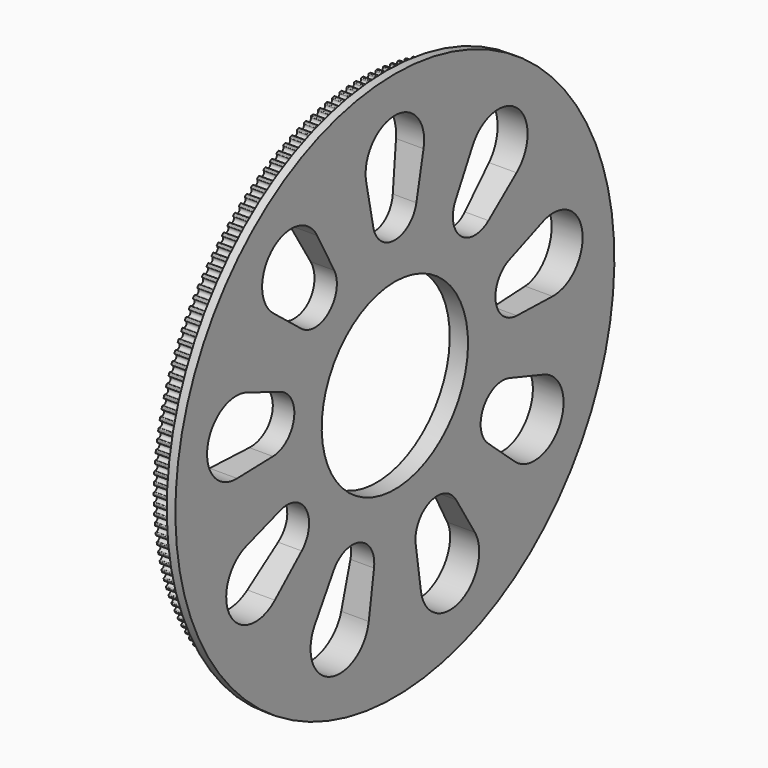
from build123d import *

# Parameters (mm, degrees)
F3_DEPTH = 17.8680288276
F5_DEPTH = 13


with BuildPart() as f1:
    # F0 (on Front) → F1 (revolve)
    with BuildSketch(Plane.XZ):
        Polygon((-4.7158686465, 139.920550967), (-17.8670288276, 139.920550967), (-10, 50), (0, 50), (0, 150), (-4.7158686465, 150), align=None)
    revolve(axis=Axis((-31.8179950118, 0, 0), (-1, 0, 0)))

    # F2 (on Right) → F3 (cut, through all)
    with BuildSketch(Plane.YZ):
        with BuildLine():
            Line((14.6969384567, 82), (19.5959179423, 106))
            ThreePointArc((19.5959179423, 106), (0, 130), (-19.5959179423, 106))
            Line((-19.5959179423, 106), (-14.6969384567, 82))
            ThreePointArc((-14.6969384567, 82), (0, 70), (14.6969384567, 82))
        make_face()
        with BuildLine():
            ThreePointArc((-53.1241425793, 93.7967242243), (-83.5623892593, 99.5857776055), (-83.1468306743, 68.6046977169))
            Line((-83.1468306743, 68.6046977169), (-63.9670920299, 53.3686343955))
            ThreePointArc((-63.9670920299, 53.3686343955), (-44.9951326781, 53.6231110183), (-41.4500759587, 72.262654276))
            Line((-41.4500759587, 72.262654276), (-53.1241425793, 93.7967242243))
        make_face()
        with BuildLine():
            ThreePointArc((-100.9868263789, 37.7049187496), (-128.0250078916, 22.5742630967), (-107.7924172597, -0.8915050842))
            Line((-107.7924172597, -0.8915050842), (-83.3063323273, -0.234508369))
            ThreePointArc((-83.3063323273, -0.234508369), (-68.9365427109, 12.1553724367), (-78.2021391667, 28.7128095064))
            Line((-78.2021391667, 28.7128095064), (-100.9868263789, 37.7049187496))
        make_face()
        with BuildLine():
            ThreePointArc((-101.5966517723, -36.0294372515), (-112.583302492, -65), (-82.00073383, -69.9705627485))
            Line((-82.00073383, -69.9705627485), (-63.665613882, -53.7279220614))
            ThreePointArc((-63.665613882, -53.7279220614), (-60.6217782649, -35), (-78.3625523387, -28.2720779386))
            Line((-78.3625523387, -28.2720779386), (-101.5966517723, -36.0294372515))
        make_face()
        with BuildLine():
            ThreePointArc((-54.6682746804, -92.9052191401), (-44.4626186323, -122.1600407022), (-17.8399957046, -106.3096164665))
            Line((-17.8399957046, -106.3096164665), (-14.2350471368, -82.0814439019))
            ThreePointArc((-14.2350471368, -82.0814439019), (-23.9414100328, -65.778483455), (-41.8562563686, -72.028145907))
            Line((-41.8562563686, -72.028145907), (-54.6682746804, -92.9052191401))
        make_face()
        with BuildLine():
            ThreePointArc((17.8399957046, -106.3096164665), (44.4626186323, -122.1600407022), (54.6682746804, -92.9052191401))
            Line((54.6682746804, -92.9052191401), (41.8562563686, -72.028145907))
            ThreePointArc((41.8562563686, -72.028145907), (23.9414100328, -65.778483455), (14.2350471368, -82.0814439019))
            Line((14.2350471368, -82.0814439019), (17.8399957046, -106.3096164665))
        make_face()
        with BuildLine():
            ThreePointArc((82.00073383, -69.9705627485), (112.583302492, -65), (101.5966517723, -36.0294372515))
            Line((101.5966517723, -36.0294372515), (78.3625523387, -28.2720779386))
            ThreePointArc((78.3625523387, -28.2720779386), (60.6217782649, -35), (63.665613882, -53.7279220614))
            Line((63.665613882, -53.7279220614), (82.00073383, -69.9705627485))
        make_face()
        with BuildLine():
            ThreePointArc((107.7924172597, -0.8915050842), (128.0250078916, 22.5742630967), (100.9868263789, 37.7049187496))
            Line((100.9868263789, 37.7049187496), (78.2021391667, 28.7128095064))
            ThreePointArc((78.2021391667, 28.7128095064), (68.9365427109, 12.1553724367), (83.3063323273, -0.234508369))
            Line((83.3063323273, -0.234508369), (107.7924172597, -0.8915050842))
        make_face()
        with BuildLine():
            Line((53.1241425793, 93.7967242243), (41.4500759587, 72.262654276))
            ThreePointArc((41.4500759587, 72.262654276), (44.9951326781, 53.6231110183), (63.9670920299, 53.3686343955))
            Line((63.9670920299, 53.3686343955), (83.1468306743, 68.6046977169))
            ThreePointArc((83.1468306743, 68.6046977169), (83.5623892593, 99.5857776055), (53.1241425793, 93.7967242243))
        make_face()
    extrude(amount=-F3_DEPTH, mode=Mode.SUBTRACT)

    # F4 (on face) → F5 (join)
    with BuildSketch(Plane(origin=(-4.7158686465, 0, 0), x_dir=(0, -1, 0), z_dir=(-1, 0, 0))):
        with BuildLine():
            ThreePointArc((4.0237123473, 142.1136204842), (2.4517908469, 140.4630035454), (0.9384326191, 142.1674742422))
            ThreePointArc((0.9384326191, 142.1674742422), (0.8241772032, 142.5169854565), (0.4885078504, 142.6671136502))
            Line((0.4885078504, 142.6671136502), (0, 142.66795))
            Line((0, 142.66795), (0, 137.7496519993))
            Line((0, 137.7496519993), (4.8044649915, 137.5818763848))
            Line((4.8044649915, 137.5818763848), (4.8073935257, 137.6657386332))
            Line((4.8073935257, 137.6657386332), (4.9790396506, 142.5810405396))
            Line((4.9790396506, 142.5810405396), (4.9790688389, 142.5818763848))
            Line((4.9790688389, 142.5818763848), (4.4908001977, 142.5972533774))
            ThreePointArc((4.4908001977, 142.5972533774), (4.1500959272, 142.4589313292), (4.0237123473, 142.1136204842))
        make_face()
        with BuildLine():
            Line((0, 137.7496519993), (0, 142.66795))
            Line((0, 142.66795), (0, 142.6687863547))
            Line((0, 142.6687863547), (-0.4885078504, 142.6671136502))
            ThreePointArc((-0.4885078504, 142.6671136502), (-0.8241772032, 142.5169854565), (-0.9384326191, 142.1674742422))
            ThreePointArc((-0.9384326191, 142.1674742422), (-2.4517908469, 140.4630035454), (-4.0237123473, 142.1136204842))
            ThreePointArc((-4.0237123473, 142.1136204842), (-4.1500959272, 142.4589313292), (-4.4908001977, 142.5972533774))
            Line((-4.4908001977, 142.5972533774), (-4.9790396506, 142.5810405396))
            Line((-4.9790396506, 142.5810405396), (-4.8073935257, 137.6657386332))
            Line((-4.8073935257, 137.6657386332), (0, 137.6657386332))
            Line((0, 137.6657386332), (0, 137.7496519993))
        make_face()
        with BuildLine():
            Line((5.467220727, 142.5631560212), (4.9790396506, 142.5810405396))
            Line((4.9790396506, 142.5810405396), (4.8073935257, 137.6657386332))
            Line((4.8073935257, 137.6657386332), (9.6030764824, 137.3303918129))
            Line((9.6030764824, 137.3303918129), (9.608929983, 137.4141007703))
            Line((9.608929983, 137.4141007703), (9.9520131083, 142.3204180443))
            Line((9.9520131083, 142.3204180443), (9.9520714495, 142.3212523616))
            Line((9.9520714495, 142.3212523616), (9.4646368976, 142.3536603168))
            ThreePointArc((9.4646368976, 142.3536603168), (9.1193128051, 142.2273129382), (8.9809550399, 141.8866231706))
            ThreePointArc((8.9809550399, 141.8866231706), (7.3523854112, 140.2918710123), (5.8994342498, 142.048118832))
            ThreePointArc((5.8994342498, 142.048118832), (5.7974462007, 142.40140459), (5.467220727, 142.5631560212))
        make_face()
        with BuildLine():
            Line((-4.8044649915, 137.5818763848), (-4.8073935257, 137.6657386332))
            Line((-4.8073935257, 137.6657386332), (-4.9790396506, 142.5810405396))
            Line((-4.9790396506, 142.5810405396), (-4.9790688389, 142.5818763848))
            Line((-4.9790688389, 142.5818763848), (-5.467220727, 142.5631560212))
            ThreePointArc((-5.467220727, 142.5631560212), (-5.7974462007, 142.40140459), (-5.8994342498, 142.048118832))
            ThreePointArc((-5.8994342498, 142.048118832), (-7.3523854112, 140.2918710123), (-8.9809550399, 141.8866231706))
            ThreePointArc((-8.9809550399, 141.8866231706), (-9.1193128051, 142.2273129382), (-9.4646368976, 142.3536603168))
            Line((-9.4646368976, 142.3536603168), (-9.9520131083, 142.3204180443))
            Line((-9.9520131083, 142.3204180443), (-9.608929983, 137.4141007703))
            Line((-9.608929983, 137.4141007703), (-4.8044649915, 137.5818763848))
        make_face()
        with BuildLine():
            Line((9.9520131083, 142.3204180443), (9.608929983, 137.4141007703))
            Line((9.608929983, 137.4141007703), (14.3899881039, 136.9115913128))
            Line((14.3899881039, 136.9115913128), (14.3987594391, 136.9950449927))
            Line((14.3987594391, 136.9950449927), (14.912861571, 141.8864000423))
            Line((14.912861571, 141.8864000423), (14.9129489939, 141.8872318154))
            Line((14.9129489939, 141.8872318154), (14.4269423954, 141.936631249))
            ThreePointArc((14.4269423954, 141.936631249), (14.077419205, 141.8224124749), (13.9272558222, 141.4867588626))
            ThreePointArc((13.9272558222, 141.4867588626), (12.2440222265, 139.9498144446), (10.8532483286, 141.7556996699))
            ThreePointArc((10.8532483286, 141.7556996699), (10.7636519031, 142.1123295473), (10.4392726374, 142.2855071467))
            Line((10.4392726374, 142.2855071467), (9.9520131083, 142.3204180443))
        make_face()
        with BuildLine():
            Line((-9.6030764824, 137.3303918129), (-9.608929983, 137.4141007703))
            Line((-9.608929983, 137.4141007703), (-9.9520131083, 142.3204180443))
            Line((-9.9520131083, 142.3204180443), (-9.9520714495, 142.3212523616))
            Line((-9.9520714495, 142.3212523616), (-10.4392726374, 142.2855071467))
            ThreePointArc((-10.4392726374, 142.2855071467), (-10.7636519031, 142.1123295473), (-10.8532483286, 141.7556996699))
            ThreePointArc((-10.8532483286, 141.7556996699), (-12.2440222265, 139.9498144446), (-13.9272558222, 141.4867588626))
            ThreePointArc((-13.9272558222, 141.4867588626), (-14.077419205, 141.8224124749), (-14.4269423954, 141.936631249))
            Line((-14.4269423954, 141.936631249), (-14.912861571, 141.8864000423))
            Line((-14.912861571, 141.8864000423), (-14.3987594391, 136.9950449927))
            Line((-14.3987594391, 136.9950449927), (-9.6030764824, 137.3303918129))
        make_face()
        with BuildLine():
            Line((14.912861571, 141.8864000423), (14.3987594391, 136.9950449927))
            Line((14.3987594391, 136.9950449927), (19.1593677415, 136.3259851282))
            Line((19.1593677415, 136.3259851282), (19.1710462249, 136.4090818552))
            Line((19.1710462249, 136.4090818552), (19.8555410091, 141.2795153178))
            Line((19.8555410091, 141.2795153178), (19.8556574072, 141.2803435332))
            Line((19.8556574072, 141.2803435332), (19.3716708861, 141.3466742597))
            ThreePointArc((19.3716708861, 141.3466742597), (19.0183744381, 141.244723248), (18.8565883886, 140.9145147333))
            ThreePointArc((18.8565883886, 140.9145147333), (17.1207415867, 139.4372505856), (15.7938393962, 141.2905730235))
            ThreePointArc((15.7938393962, 141.2905730235), (15.7167437536, 141.6501125218), (15.398605902, 141.8345052992))
            Line((15.398605902, 141.8345052992), (14.912861571, 141.8864000423))
        make_face()
        with BuildLine():
            Line((-14.3899881039, 136.9115913128), (-14.3987594391, 136.9950449927))
            Line((-14.3987594391, 136.9950449927), (-14.912861571, 141.8864000423))
            Line((-14.912861571, 141.8864000423), (-14.9129489939, 141.8872318154))
            Line((-14.9129489939, 141.8872318154), (-15.398605902, 141.8345052992))
            ThreePointArc((-15.398605902, 141.8345052992), (-15.7167437536, 141.6501125218), (-15.7938393962, 141.2905730235))
            ThreePointArc((-15.7938393962, 141.2905730235), (-17.1207415867, 139.4372505856), (-18.8565883886, 140.9145147333))
            ThreePointArc((-18.8565883886, 140.9145147333), (-19.0183744381, 141.244723248), (-19.3716708861, 141.3466742597))
            Line((-19.3716708861, 141.3466742597), (-19.8555410091, 141.2795153178))
            Line((-19.8555410091, 141.2795153178), (-19.1710462249, 136.4090818552))
            Line((-19.1710462249, 136.4090818552), (-14.3899881039, 136.9115913128))
        make_face()
        with BuildLine():
            Line((19.8555410091, 141.2795153178), (19.1710462249, 136.4090818552))
            Line((19.1710462249, 136.4090818552), (23.9054046408, 135.5742867301))
            Line((23.9054046408, 135.5742867301), (23.9199760439, 135.6569252637))
            Line((23.9199760439, 135.6569252637), (24.774029529, 140.5005032664))
            Line((24.774029529, 140.5005032664), (24.7741747604, 140.5013269149))
            Line((24.7741747604, 140.5013269149), (24.2927979798, 140.5845081206))
            ThreePointArc((24.2927979798, 140.5845081206), (23.9361587115, 140.4949490829), (23.7629471067, 140.170587974))
            ThreePointArc((23.7629471067, 140.170587974), (21.9766019605, 138.7548039155), (20.7151881033, 140.653305578))
            ThreePointArc((20.7151881033, 140.653305578), (20.6506871728, 141.0153166537), (20.3391783373, 141.2106999549))
            Line((20.3391783373, 141.2106999549), (19.8555410091, 141.2795153178))
        make_face()
        with BuildLine():
            Line((-19.1593677415, 136.3259851282), (-19.1710462249, 136.4090818552))
            Line((-19.1710462249, 136.4090818552), (-19.8555410091, 141.2795153178))
            Line((-19.8555410091, 141.2795153178), (-19.8556574072, 141.2803435332))
            Line((-19.8556574072, 141.2803435332), (-20.3391783373, 141.2106999549))
            ThreePointArc((-20.3391783373, 141.2106999549), (-20.6506871728, 141.0153166537), (-20.7151881033, 140.653305578))
            ThreePointArc((-20.7151881033, 140.653305578), (-21.9766019605, 138.7548039155), (-23.7629471067, 140.170587974))
            ThreePointArc((-23.7629471067, 140.170587974), (-23.9361587115, 140.4949490829), (-24.2927979798, 140.5845081206))
            Line((-24.2927979798, 140.5845081206), (-24.774029529, 140.5005032664))
            Line((-24.774029529, 140.5005032664), (-23.9199760439, 135.6569252637))
            Line((-23.9199760439, 135.6569252637), (-19.1593677415, 136.3259851282))
        make_face()
        with BuildLine():
            Line((24.774029529, 140.5005032664), (23.9199760439, 135.6569252637))
            Line((23.9199760439, 135.6569252637), (28.6223164869, 134.6574119473))
            Line((28.6223164869, 134.6574119473), (28.6397630567, 134.7394916051))
            Line((28.6397630567, 134.7394916051), (29.66233471, 139.5503129941))
            Line((29.66233471, 139.5503129941), (29.6625085979, 139.5511310724))
            Line((29.6625085979, 139.5511310724), (29.1843280413, 139.6510614137))
            ThreePointArc((29.1843280413, 139.6510614137), (28.8247804626, 139.5740034639), (28.6403543342, 139.2558849449))
            ThreePointArc((28.6403543342, 139.2558849449), (26.8056872301, 137.9033058903), (25.6112985446, 139.8446737457))
            ThreePointArc((25.6112985446, 139.8446737457), (25.5594709107, 140.208715344), (25.2549706169, 140.4148511246))
            Line((25.2549706169, 140.4148511246), (24.774029529, 140.5005032664))
        make_face()
        with BuildLine():
            Line((-23.9054046408, 135.5742867301), (-23.9199760439, 135.6569252637))
            Line((-23.9199760439, 135.6569252637), (-24.774029529, 140.5005032664))
            Line((-24.774029529, 140.5005032664), (-24.7741747604, 140.5013269149))
            Line((-24.7741747604, 140.5013269149), (-25.2549706169, 140.4148511246))
            ThreePointArc((-25.2549706169, 140.4148511246), (-25.5594709107, 140.208715344), (-25.6112985446, 139.8446737457))
            ThreePointArc((-25.6112985446, 139.8446737457), (-26.8056872301, 137.9033058903), (-28.6403543342, 139.2558849449))
            ThreePointArc((-28.6403543342, 139.2558849449), (-28.8247804626, 139.5740034639), (-29.1843280413, 139.6510614137))
            Line((-29.1843280413, 139.6510614137), (-29.66233471, 139.5503129941))
            Line((-29.66233471, 139.5503129941), (-28.6397630567, 134.7394916051))
            Line((-28.6397630567, 134.7394916051), (-23.9054046408, 135.5742867301))
        make_face()
        with BuildLine():
            Line((29.66233471, 139.5503129941), (28.6397630567, 134.7394916051))
            Line((28.6397630567, 134.7394916051), (33.3043564493, 133.5764778504))
            Line((33.3043564493, 133.5764778504), (33.3246569299, 133.6578986309))
            Line((33.3246569299, 133.6578986309), (34.5145009053, 138.4301021616))
            Line((34.5145009053, 138.4301021616), (34.5147032378, 138.4309136729))
            Line((34.5147032378, 138.4309136729), (34.0403014945, 138.5474714001))
            ThreePointArc((34.0403014945, 138.5474714001), (33.6782836588, 138.4830084215), (33.4828677016, 138.1715200707))
            ThreePointArc((33.4828677016, 138.1715200707), (31.6021138989, 136.8837939293), (30.4762055638, 138.8656627198))
            ThreePointArc((30.4762055638, 138.8656627198), (30.4371143704, 139.2312913122), (30.1399936049, 139.4479284274))
            Line((30.1399936049, 139.4479284274), (29.66233471, 139.5503129941))
        make_face()
        with BuildLine():
            Line((-28.6223164869, 134.6574119473), (-28.6397630567, 134.7394916051))
            Line((-28.6397630567, 134.7394916051), (-29.66233471, 139.5503129941))
            Line((-29.66233471, 139.5503129941), (-29.6625085979, 139.5511310724))
            Line((-29.6625085979, 139.5511310724), (-30.1399936049, 139.4479284274))
            ThreePointArc((-30.1399936049, 139.4479284274), (-30.4371143704, 139.2312913122), (-30.4762055638, 138.8656627198))
            ThreePointArc((-30.4762055638, 138.8656627198), (-31.6021138989, 136.8837939293), (-33.4828677016, 138.1715200707))
            ThreePointArc((-33.4828677016, 138.1715200707), (-33.6782836588, 138.4830084215), (-34.0403014945, 138.5474714001))
            Line((-34.0403014945, 138.5474714001), (-34.5145009053, 138.4301021616))
            Line((-34.5145009053, 138.4301021616), (-33.3246569299, 133.6578986309))
            Line((-33.3246569299, 133.6578986309), (-28.6223164869, 134.6574119473))
        make_face()
        with BuildLine():
            Line((34.5145009053, 138.4301021616), (33.3246569299, 133.6578986309))
            Line((33.3246569299, 133.6578986309), (37.9458201834, 132.3328013911))
            Line((37.9458201834, 132.3328013911), (37.9689498418, 132.4134640958))
            Line((37.9689498418, 132.4134640958), (39.3246164978, 137.141235573))
            Line((39.3246164978, 137.141235573), (39.3248470284, 137.1420395288))
            Line((39.3248470284, 137.1420395288), (38.8548020838, 137.2750826342))
            ThreePointArc((38.8548020838, 137.2750826342), (38.4907550541, 137.2232931649), (38.2845873524, 136.918814483))
            ThreePointArc((38.2845873524, 136.918814483), (36.3600382598, 135.6975101507), (35.3039820209, 137.7174652745))
            ThreePointArc((35.3039820209, 137.7174652745), (35.2776748948, 138.0842353988), (34.9882956535, 138.3111099097))
            Line((34.9882956535, 138.3111099097), (34.5145009053, 138.4301021616))
        make_face()
        with BuildLine():
            Line((-33.3043564493, 133.5764778504), (-33.3246569299, 133.6578986309))
            Line((-33.3246569299, 133.6578986309), (-34.5145009053, 138.4301021616))
            Line((-34.5145009053, 138.4301021616), (-34.5147032378, 138.4309136729))
            Line((-34.5147032378, 138.4309136729), (-34.9882956535, 138.3111099097))
            ThreePointArc((-34.9882956535, 138.3111099097), (-35.2776748948, 138.0842353988), (-35.3039820209, 137.7174652745))
            ThreePointArc((-35.3039820209, 137.7174652745), (-36.3600382598, 135.6975101507), (-38.2845873524, 136.918814483))
            ThreePointArc((-38.2845873524, 136.918814483), (-38.4907550541, 137.2232931649), (-38.8548020838, 137.2750826342))
            Line((-38.8548020838, 137.2750826342), (-39.3246164978, 137.141235573))
            Line((-39.3246164978, 137.141235573), (-37.9689498418, 132.4134640958))
            Line((-37.9689498418, 132.4134640958), (-33.3043564493, 133.5764778504))
        make_face()
        with BuildLine():
            Line((39.3246164978, 137.141235573), (37.9689498418, 132.4134640958))
            Line((37.9689498418, 132.4134640958), (42.5410527808, 130.9278977977))
            Line((42.5410527808, 130.9278977977), (42.566983437, 131.0077041513))
            Line((42.566983437, 131.0077041513), (44.0868211026, 135.685283514))
            Line((44.0868211026, 135.685283514), (44.0870795504, 135.6860789345))
            Line((44.0870795504, 135.6860789345), (43.6219640819, 135.8354453257))
            ThreePointArc((43.6219640819, 135.8354453257), (43.2563313934, 135.7963924633), (43.0396631307, 135.4992944106))
            ThreePointArc((43.0396631307, 135.4992944106), (41.073663515, 134.3458998586), (40.0887460142, 136.4014803116))
            ThreePointArc((40.0887460142, 136.4014803116), (40.0752550064, 136.7689451149), (39.7939698534, 137.0057806098))
            Line((39.7939698534, 137.0057806098), (39.3246164978, 137.141235573))
        make_face()
        with BuildLine():
            Line((-37.9458201834, 132.3328013911), (-37.9689498418, 132.4134640958))
            Line((-37.9689498418, 132.4134640958), (-39.3246164978, 137.141235573))
            Line((-39.3246164978, 137.141235573), (-39.3248470284, 137.1420395288))
            Line((-39.3248470284, 137.1420395288), (-39.7939698534, 137.0057806098))
            ThreePointArc((-39.7939698534, 137.0057806098), (-40.0752550064, 136.7689451149), (-40.0887460142, 136.4014803116))
            ThreePointArc((-40.0887460142, 136.4014803116), (-41.073663515, 134.3458998586), (-43.0396631307, 135.4992944106))
            ThreePointArc((-43.0396631307, 135.4992944106), (-43.2563313934, 135.7963924633), (-43.6219640819, 135.8354453257))
            Line((-43.6219640819, 135.8354453257), (-44.0868211026, 135.685283514))
            Line((-44.0868211026, 135.685283514), (-42.566983437, 131.0077041513))
            Line((-42.566983437, 131.0077041513), (-37.9458201834, 132.3328013911))
        make_face()
        with BuildLine():
            Line((44.0868211026, 135.685283514), (42.566983437, 131.0077041513))
            Line((42.566983437, 131.0077041513), (47.0844556584, 129.3634787287))
            Line((47.0844556584, 129.3634787287), (47.1131557199, 129.4423314996))
            Line((47.1131557199, 129.4423314996), (48.795312707, 134.0640198377))
            Line((48.795312707, 134.0640198377), (48.7955987571, 134.064805754))
            Line((48.7955987571, 134.064805754), (48.3359794363, 134.2303134509))
            ThreePointArc((48.3359794363, 134.2303134509), (47.9692065561, 134.2040447753), (47.7423017093, 133.91468932))
            ThreePointArc((47.7423017093, 133.91468932), (45.737246838, 132.8306097819), (44.8246680456, 134.9193111559))
            ThreePointArc((44.8246680456, 134.9193111559), (44.8240095929, 135.2870229389), (44.5511612308, 135.5335308704))
            Line((44.5511612308, 135.5335308704), (44.0868211026, 135.685283514))
        make_face()
        with BuildLine():
            Line((-42.5410527808, 130.9278977977), (-42.566983437, 131.0077041513))
            Line((-42.566983437, 131.0077041513), (-44.0868211026, 135.685283514))
            Line((-44.0868211026, 135.685283514), (-44.0870795504, 135.6860789345))
            Line((-44.0870795504, 135.6860789345), (-44.5511612308, 135.5335308704))
            ThreePointArc((-44.5511612308, 135.5335308704), (-44.8240095929, 135.2870229389), (-44.8246680456, 134.9193111559))
            ThreePointArc((-44.8246680456, 134.9193111559), (-45.737246838, 132.8306097819), (-47.7423017093, 133.91468932))
            ThreePointArc((-47.7423017093, 133.91468932), (-47.9692065561, 134.2040447753), (-48.3359794363, 134.2303134509))
            Line((-48.3359794363, 134.2303134509), (-48.795312707, 134.0640198377))
            Line((-48.795312707, 134.0640198377), (-47.1131557199, 129.4423314996))
            Line((-47.1131557199, 129.4423314996), (-42.5410527808, 130.9278977977))
        make_face()
        with BuildLine():
            Line((48.795312707, 134.0640198377), (47.1131557199, 129.4423314996))
            Line((47.1131557199, 129.4423314996), (51.5704933795, 127.6414501877))
            Line((51.5704933795, 127.6414501877), (51.6019278797, 127.719253306))
            Line((51.6019278797, 127.719253306), (53.4443547391, 132.2794198041))
            Line((53.4443547391, 132.2794198041), (53.4446680431, 132.2801952587))
            Line((53.4446680431, 132.2801952587), (52.9911048452, 132.4616426158))
            ThreePointArc((52.9911048452, 132.4616426158), (52.6236386296, 132.4481901312), (52.3867736474, 132.1669298084))
            ThreePointArc((52.3867736474, 132.1669298084), (50.3451063711, 131.1534860682), (49.5059781238, 133.2727636023))
            ThreePointArc((49.5059781238, 133.2727636023), (49.5181530283, 133.6402743649), (49.2540738808, 133.8961544009))
            Line((49.2540738808, 133.8961544009), (48.795312707, 134.0640198377))
        make_face()
        with BuildLine():
            Line((-47.0844556584, 129.3634787287), (-47.1131557199, 129.4423314996))
            Line((-47.1131557199, 129.4423314996), (-48.795312707, 134.0640198377))
            Line((-48.795312707, 134.0640198377), (-48.7955987571, 134.064805754))
            Line((-48.7955987571, 134.064805754), (-49.2540738808, 133.8961544009))
            ThreePointArc((-49.2540738808, 133.8961544009), (-49.5181530283, 133.6402743649), (-49.5059781238, 133.2727636023))
            ThreePointArc((-49.5059781238, 133.2727636023), (-50.3451063711, 131.1534860682), (-52.3867736474, 132.1669298084))
            ThreePointArc((-52.3867736474, 132.1669298084), (-52.6236386296, 132.4481901312), (-52.9911048452, 132.4616426158))
            Line((-52.9911048452, 132.4616426158), (-53.4443547391, 132.2794198041))
            Line((-53.4443547391, 132.2794198041), (-51.6019278797, 127.719253306))
            Line((-51.6019278797, 127.719253306), (-47.0844556584, 129.3634787287))
        make_face()
        with BuildLine():
            Line((53.4443547391, 132.2794198041), (51.6019278797, 127.719253306))
            Line((51.6019278797, 127.719253306), (55.9937003982, 125.7639102014))
            Line((55.9937003982, 125.7639102014), (56.0278310391, 125.8405688758))
            Line((56.0278310391, 125.8405688758), (58.0282830575, 130.3336576737))
            Line((58.0282830575, 130.3336576737), (58.0286232336, 130.3344217217))
            Line((58.0286232336, 130.3344217217), (57.5816687556, 130.5315876733))
            ThreePointArc((57.5816687556, 130.5315876733), (57.2139569055, 130.5309677696), (56.9674203714, 130.2581452517))
            ThreePointArc((56.9674203714, 130.2581452517), (54.8916281471, 129.3165720344), (54.1269727934, 131.4638437153))
            ThreePointArc((54.1269727934, 131.4638437153), (54.1519662219, 131.8307057023), (53.8969780287, 132.0956460924))
            Line((53.8969780287, 132.0956460924), (53.4443547391, 132.2794198041))
        make_face()
        with BuildLine():
            Line((-51.5704933795, 127.6414501877), (-51.6019278797, 127.719253306))
            Line((-51.6019278797, 127.719253306), (-53.4443547391, 132.2794198041))
            Line((-53.4443547391, 132.2794198041), (-53.4446680431, 132.2801952587))
            Line((-53.4446680431, 132.2801952587), (-53.8969780287, 132.0956460924))
            ThreePointArc((-53.8969780287, 132.0956460924), (-54.1519662219, 131.8307057023), (-54.1269727934, 131.4638437153))
            ThreePointArc((-54.1269727934, 131.4638437153), (-54.8916281471, 129.3165720344), (-56.9674203714, 130.2581452517))
            ThreePointArc((-56.9674203714, 130.2581452517), (-57.2139569055, 130.5309677696), (-57.5816687556, 130.5315876733))
            Line((-57.5816687556, 130.5315876733), (-58.0282830575, 130.3336576737))
            Line((-58.0282830575, 130.3336576737), (-56.0278310391, 125.8405688758))
            Line((-56.0278310391, 125.8405688758), (-51.5704933795, 127.6414501877))
        make_face()
        with BuildLine():
            Line((58.0282830575, 130.3336576737), (56.0278310391, 125.8405688758))
            Line((56.0278310391, 125.8405688758), (60.3486877182, 123.7331462629))
            Line((60.3486877182, 123.7331462629), (60.3854729167, 123.8085670968))
            Line((60.3854729167, 123.8085670968), (62.5415128515, 128.2291040577))
            Line((62.5415128515, 128.2291040577), (62.5418794853, 128.2298557683))
            Line((62.5418794853, 128.2298557683), (62.1020782724, 128.4425000981))
            ThreePointArc((62.1020782724, 128.4425000981), (61.7345687881, 128.4547135305), (61.4786610688, 128.1906612096))
            ThreePointArc((61.4786610688, 128.1906612096), (59.3712729297, 127.3221056772), (58.6820220843, 129.4947553852))
            ThreePointArc((58.6820220843, 129.4947553852), (58.7198035862, 129.8605216317), (58.4742170112, 130.1341995869))
            Line((58.4742170112, 130.1341995869), (58.0282830575, 130.3336576737))
        make_face()
        with BuildLine():
            Line((-55.9937003982, 125.7639102014), (-56.0278310391, 125.8405688758))
            Line((-56.0278310391, 125.8405688758), (-58.0282830575, 130.3336576737))
            Line((-58.0282830575, 130.3336576737), (-58.0286232336, 130.3344217217))
            Line((-58.0286232336, 130.3344217217), (-58.4742170112, 130.1341995869))
            ThreePointArc((-58.4742170112, 130.1341995869), (-58.7198035862, 129.8605216317), (-58.6820220843, 129.4947553852))
            ThreePointArc((-58.6820220843, 129.4947553852), (-59.3712729297, 127.3221056772), (-61.4786610688, 128.1906612096))
            ThreePointArc((-61.4786610688, 128.1906612096), (-61.7345687881, 128.4547135305), (-62.1020782724, 128.4425000981))
            Line((-62.1020782724, 128.4425000981), (-62.5415128515, 128.2291040577))
            Line((-62.5415128515, 128.2291040577), (-60.3854729167, 123.8085670968))
            Line((-60.3854729167, 123.8085670968), (-55.9937003982, 125.7639102014))
        make_face()
        with BuildLine():
            Line((62.5415128515, 128.2291040577), (60.3854729167, 123.8085670968))
            Line((60.3854729167, 123.8085670968), (64.6301494582, 121.5516325453))
            Line((64.6301494582, 121.5516325453), (64.6695443973, 121.62572365))
            Line((64.6695443973, 121.62572365), (66.978545446, 125.9683230306))
            Line((66.978545446, 125.9683230306), (66.9789380907, 125.969061488))
            Line((66.9789380907, 125.969061488), (66.5468259729, 126.1969251216))
            ThreePointArc((66.5468259729, 126.1969251216), (66.1799666081, 126.2219570099), (65.9149994877, 125.9669965932))
            ThreePointArc((65.9149994877, 125.9669965932), (63.7785829616, 125.1725169467), (63.1655763705, 127.3678976428))
            ThreePointArc((63.1655763705, 127.3678976428), (63.2160999148, 127.732122519), (62.9802141675, 128.0142046049))
            Line((62.9802141675, 128.0142046049), (62.5415128515, 128.2291040577))
        make_face()
        with BuildLine():
            Line((-60.3486877182, 123.7331462629), (-60.3854729167, 123.8085670968))
            Line((-60.3854729167, 123.8085670968), (-62.5415128515, 128.2291040577))
            Line((-62.5415128515, 128.2291040577), (-62.5418794853, 128.2298557683))
            Line((-62.5418794853, 128.2298557683), (-62.9802141675, 128.0142046049))
            ThreePointArc((-62.9802141675, 128.0142046049), (-63.2160999148, 127.732122519), (-63.1655763705, 127.3678976428))
            ThreePointArc((-63.1655763705, 127.3678976428), (-63.7785829616, 125.1725169467), (-65.9149994877, 125.9669965932))
            ThreePointArc((-65.9149994877, 125.9669965932), (-66.1799666081, 126.2219570099), (-66.5468259729, 126.1969251216))
            Line((-66.5468259729, 126.1969251216), (-66.978545446, 125.9683230306))
            Line((-66.978545446, 125.9683230306), (-64.6695443973, 121.62572365))
            Line((-64.6695443973, 121.62572365), (-60.3486877182, 123.7331462629))
        make_face()
        with BuildLine():
            Line((66.978545446, 125.9683230306), (64.6695443973, 121.62572365))
            Line((64.6695443973, 121.62572365), (68.8328693166, 119.2220268871))
            Line((68.8328693166, 119.2220268871), (68.8748259997, 119.2946979939))
            Line((68.8748259997, 119.2946979939), (71.333975, 123.5540690058))
            Line((71.333975, 123.5540690058), (71.3343931773, 123.5547933103))
            Line((71.3343931773, 123.5547933103), (70.9104966167, 123.7975986309))
            ThreePointArc((70.9104966167, 123.7975986309), (70.544734333, 123.8354184777), (70.2710306332, 123.5898605951))
            ThreePointArc((70.2710306332, 123.5898605951), (68.1081886145, 122.8704247857), (67.5721731318, 125.0858617367))
            ThreePointArc((67.5721731318, 125.0858617367), (67.6353771635, 125.4481014907), (67.4094796341, 125.7382440336))
            Line((67.4094796341, 125.7382440336), (66.978545446, 125.9683230306))
        make_face()
        with BuildLine():
            Line((-64.6301494582, 121.5516325453), (-64.6695443973, 121.62572365))
            Line((-64.6695443973, 121.62572365), (-66.978545446, 125.9683230306))
            Line((-66.978545446, 125.9683230306), (-66.9789380907, 125.969061488))
            Line((-66.9789380907, 125.969061488), (-67.4094796341, 125.7382440336))
            ThreePointArc((-67.4094796341, 125.7382440336), (-67.6353771635, 125.4481014907), (-67.5721731318, 125.0858617367))
            ThreePointArc((-67.5721731318, 125.0858617367), (-68.1081886145, 122.8704247857), (-70.2710306332, 123.5898605951))
            ThreePointArc((-70.2710306332, 123.5898605951), (-70.544734333, 123.8354184777), (-70.9104966167, 123.7975986309))
            Line((-70.9104966167, 123.7975986309), (-71.333975, 123.5540690058))
            Line((-71.333975, 123.5540690058), (-68.8748259997, 119.2946979939))
            Line((-68.8748259997, 119.2946979939), (-64.6301494582, 121.5516325453))
        make_face()
        with BuildLine():
            Line((71.333975, 123.5540690058), (68.8748259997, 119.2946979939))
            Line((68.8748259997, 119.2946979939), (72.9517269266, 116.7471675539))
            Line((72.9517269266, 116.7471675539), (72.9961942359, 116.8183301242))
            Line((72.9961942359, 116.8183301242), (75.6024950937, 120.98928338))
            Line((75.6024950937, 120.98928338), (75.6029382941, 120.989992649))
            Line((75.6029382941, 120.989992649), (75.1877737433, 121.2474438359))
            ThreePointArc((75.1877737433, 121.2474438359), (74.8235541657, 121.2980055634), (74.5414473523, 121.0621493895))
            ThreePointArc((74.5414473523, 121.0621493895), (72.3548149309, 120.4186339388), (71.8964436089, 122.6514279761))
            ThreePointArc((71.8964436089, 122.6514279761), (71.9722511235, 123.0112412745), (71.7566170335, 123.3090907805))
            Line((71.7566170335, 123.3090907805), (71.333975, 123.5540690058))
        make_face()
        with BuildLine():
            Line((-68.8328693166, 119.2220268871), (-68.8748259997, 119.2946979939))
            Line((-68.8748259997, 119.2946979939), (-71.333975, 123.5540690058))
            Line((-71.333975, 123.5540690058), (-71.3343931773, 123.5547933103))
            Line((-71.3343931773, 123.5547933103), (-71.7566170335, 123.3090907805))
            ThreePointArc((-71.7566170335, 123.3090907805), (-71.9722511235, 123.0112412745), (-71.8964436089, 122.6514279761))
            ThreePointArc((-71.8964436089, 122.6514279761), (-72.3548149309, 120.4186339388), (-74.5414473523, 121.0621493895))
            ThreePointArc((-74.5414473523, 121.0621493895), (-74.8235541657, 121.2980055634), (-75.1877737433, 121.2474438359))
            Line((-75.1877737433, 121.2474438359), (-75.6024950937, 120.98928338))
            Line((-75.6024950937, 120.98928338), (-72.9961942359, 116.8183301242))
            Line((-72.9961942359, 116.8183301242), (-68.8328693166, 119.2220268871))
        make_face()
        with BuildLine():
            Line((75.6024950937, 120.98928338), (72.9961942359, 116.8183301242))
            Line((72.9961942359, 116.8183301242), (76.9817040947, 114.1300697805))
            Line((76.9817040947, 114.1300697805), (77.0286278536, 114.1996371138))
            Line((77.0286278536, 114.1996371138), (79.7789051927, 118.2770909494))
            Line((79.7789051927, 118.2770909494), (79.7793728763, 118.2777843189))
            Line((79.7793728763, 118.2777843189), (79.3734461494, 118.5495677073))
            ThreePointArc((79.3734461494, 118.5495677073), (79.0112130234, 118.6128097139), (78.7210468001, 118.386942603))
            ThreePointArc((78.7210468001, 118.386942603), (76.5132880507, 117.8201315355), (76.1331193443, 120.0675623434))
            ThreePointArc((76.1331193443, 120.0675623434), (76.2214379819, 120.4245108092), (76.0163300483, 120.7297043945))
            Line((76.0163300483, 120.7297043945), (75.6024950937, 120.98928338))
        make_face()
        with BuildLine():
            Line((-72.9517269266, 116.7471675539), (-72.9961942359, 116.8183301242))
            Line((-72.9961942359, 116.8183301242), (-75.6024950937, 120.98928338))
            Line((-75.6024950937, 120.98928338), (-75.6029382941, 120.989992649))
            Line((-75.6029382941, 120.989992649), (-76.0163300483, 120.7297043945))
            ThreePointArc((-76.0163300483, 120.7297043945), (-76.2214379819, 120.4245108092), (-76.1331193443, 120.0675623434))
            ThreePointArc((-76.1331193443, 120.0675623434), (-76.5132880507, 117.8201315355), (-78.7210468001, 118.386942603))
            ThreePointArc((-78.7210468001, 118.386942603), (-79.0112130234, 118.6128097139), (-79.3734461494, 118.5495677073))
            Line((-79.3734461494, 118.5495677073), (-79.7789051927, 118.2770909494))
            Line((-79.7789051927, 118.2770909494), (-77.0286278536, 114.1996371138))
            Line((-77.0286278536, 114.1996371138), (-72.9517269266, 116.7471675539))
        make_face()
        with BuildLine():
            Line((79.7789051927, 118.2770909494), (77.0286278536, 114.1996371138))
            Line((77.0286278536, 114.1996371138), (80.9178909145, 111.3739220974))
            Line((80.9178909145, 111.3739220974), (80.9672139536, 111.4418094367))
            Line((80.9672139536, 111.4418094367), (83.8581169848, 115.4207961026))
            Line((83.8581169848, 115.4207961026), (83.8586085818, 115.4214727278))
            Line((83.8586085818, 115.4214727278), (83.4624142378, 115.7072571916))
            ThreePointArc((83.4624142378, 115.7072571916), (83.1026088887, 115.7831024267), (82.8047367783, 115.567499563))
            ThreePointArc((82.8047367783, 115.567499563), (80.5785415149, 115.0780834507), (80.2770386011, 117.337412881))
            ThreePointArc((80.2770386011, 117.337412881), (80.3777607592, 117.6910616274), (80.1834288743, 118.0032274608))
            Line((80.1834288743, 118.0032274608), (79.7789051927, 118.2770909494))
        make_face()
        with BuildLine():
            Line((-76.9817040947, 114.1300697805), (-77.0286278536, 114.1996371138))
            Line((-77.0286278536, 114.1996371138), (-79.7789051927, 118.2770909494))
            Line((-79.7789051927, 118.2770909494), (-79.7793728763, 118.2777843189))
            Line((-79.7793728763, 118.2777843189), (-80.1834288743, 118.0032274608))
            ThreePointArc((-80.1834288743, 118.0032274608), (-80.3777607592, 117.6910616274), (-80.2770386011, 117.337412881))
            ThreePointArc((-80.2770386011, 117.337412881), (-80.5785415149, 115.0780834507), (-82.8047367783, 115.567499563))
            ThreePointArc((-82.8047367783, 115.567499563), (-83.1026088887, 115.7831024267), (-83.4624142378, 115.7072571916))
            Line((-83.4624142378, 115.7072571916), (-83.8581169848, 115.4207961026))
            Line((-83.8581169848, 115.4207961026), (-80.9672139536, 111.4418094367))
            Line((-80.9672139536, 111.4418094367), (-76.9817040947, 114.1300697805))
        make_face()
        with BuildLine():
            Line((83.8581169848, 115.4207961026), (80.9672139536, 111.4418094367))
            Line((80.9672139536, 111.4418094367), (84.7554917487, 108.4820824462))
            Line((84.7554917487, 108.4820824462), (84.8071539755, 108.5482070811))
            Line((84.8071539755, 108.5482070811), (87.8351605787, 112.423878795))
            Line((87.8351605787, 112.423878795), (87.8356754901, 112.4245378515))
            Line((87.83567549, 112.4245378515), (87.449696231, 112.7239752063))
            ThreePointArc((87.449696231, 112.7239752063), (87.0927570261, 112.8123312642), (86.7875419399, 112.6072553267))
            ThreePointArc((86.7875419399, 112.6072553267), (84.5456224385, 112.1958304477), (84.3231526521, 114.4643058555))
            ThreePointArc((84.3231526521, 114.4643058555), (84.4361556163, 114.814224016), (84.2528365436, 115.1329817713))
            Line((84.2528365436, 115.1329817713), (83.8581169848, 115.4207961026))
        make_face()
        with BuildLine():
            Line((-80.9178909145, 111.3739220974), (-80.9672139536, 111.4418094367))
            Line((-80.9672139536, 111.4418094367), (-83.8581169848, 115.4207961026))
            Line((-83.8581169848, 115.4207961026), (-83.8586085818, 115.4214727278))
            Line((-83.8586085818, 115.4214727278), (-84.2528365436, 115.1329817713))
            ThreePointArc((-84.2528365436, 115.1329817713), (-84.4361556163, 114.814224016), (-84.3231526521, 114.4643058555))
            ThreePointArc((-84.3231526521, 114.4643058555), (-84.5456224385, 112.1958304477), (-86.7875419399, 112.6072553267))
            ThreePointArc((-86.7875419399, 112.6072553267), (-87.0927570261, 112.8123312642), (-87.449696231, 112.7239752063))
            Line((-87.449696231, 112.7239752063), (-87.8351605787, 112.423878795))
            Line((-87.8351605787, 112.423878795), (-84.8071539755, 108.5482070811))
            Line((-84.8071539755, 108.5482070811), (-80.9178909145, 111.3739220974))
        make_face()
        with BuildLine():
            Line((87.8351605787, 112.423878795), (84.8071539755, 108.5482070811))
            Line((84.8071539755, 108.5482070811), (88.4898310718, 105.4580740878))
            Line((88.4898310718, 105.4580740878), (88.5437695438, 105.5223554557))
            Line((88.5437695438, 105.5223554557), (91.7051905594, 109.2899903087))
            Line((91.7051905594, 109.2899903087), (91.7057281578, 109.2906309935))
            Line((91.7057281578, 109.2906309935), (91.3304342399, 109.6033564211))
            ThreePointArc((91.3304342399, 109.6033564211), (90.9767960546, 109.7041156534), (90.6646098502, 109.5098164955))
            ThreePointArc((90.6646098502, 109.5098164955), (88.4096975444, 109.1768841077), (88.2665319306, 111.4517417052))
            ThreePointArc((88.2665319306, 111.4517417052), (88.3916780241, 111.7975029584), (88.2195951097, 112.1224642785))
            Line((88.2195951097, 112.1224642785), (87.8351605787, 112.423878795))
        make_face()
        with BuildLine():
            Line((-84.7554917487, 108.4820824462), (-84.8071539755, 108.5482070811))
            Line((-84.8071539755, 108.5482070811), (-87.8351605787, 112.423878795))
            Line((-87.8351605787, 112.423878795), (-87.83567549, 112.4245378515))
            Line((-87.8356754901, 112.4245378515), (-88.2195951097, 112.1224642785))
            ThreePointArc((-88.2195951097, 112.1224642785), (-88.3916780241, 111.7975029584), (-88.2665319306, 111.4517417052))
            ThreePointArc((-88.2665319306, 111.4517417052), (-88.4096975444, 109.1768841077), (-90.6646098502, 109.5098164955))
            ThreePointArc((-90.6646098502, 109.5098164955), (-90.9767960546, 109.7041156534), (-91.3304342399, 109.6033564211))
            Line((-91.3304342399, 109.6033564211), (-91.7051905594, 109.2899903087))
            Line((-91.7051905594, 109.2899903087), (-88.5437695438, 105.5223554557))
            Line((-88.5437695438, 105.5223554557), (-84.7554917487, 108.4820824462))
        make_face()
        with BuildLine():
            Line((91.7051905594, 109.2899903087), (88.5437695438, 105.5223554557))
            Line((88.5437695438, 105.5223554557), (92.1163591665, 102.3055813108))
            Line((92.1163591665, 102.3055813108), (92.172508168, 102.3679410946))
            Line((92.172508168, 102.3679410946), (95.4634918915, 106.022948804))
            Line((95.4634918915, 106.022948804), (95.464051522, 106.0235703366))
            Line((95.464051522, 106.0235703366), (95.099900183, 106.3492028291))
            ThreePointArc((95.099900183, 106.3492028291), (94.7499938711, 106.4622424764), (94.4312168993, 106.2789568217))
            ThreePointArc((94.4312168993, 106.2789568217), (92.1660590523, 106.0249225518), (92.1023720364, 108.3033907754))
            ThreePointArc((92.1023720364, 108.3033907754), (92.239508788, 108.6445738646), (92.0788716883, 108.9753428341))
            Line((92.0788716883, 108.9753428341), (91.7051905594, 109.2899903087))
        make_face()
        with BuildLine():
            Line((-88.4898310718, 105.4580740878), (-88.5437695438, 105.5223554557))
            Line((-88.5437695438, 105.5223554557), (-91.7051905594, 109.2899903087))
            Line((-91.7051905594, 109.2899903087), (-91.7057281578, 109.2906309935))
            Line((-91.7057281578, 109.2906309935), (-92.0788716883, 108.9753428341))
            ThreePointArc((-92.0788716883, 108.9753428341), (-92.239508788, 108.6445738646), (-92.1023720364, 108.3033907754))
            ThreePointArc((-92.1023720364, 108.3033907754), (-92.1660590523, 106.0249225518), (-94.4312168993, 106.2789568217))
            ThreePointArc((-94.4312168993, 106.2789568217), (-94.7499938711, 106.4622424764), (-95.099900183, 106.3492028291))
            Line((-95.099900183, 106.3492028291), (-95.4634918915, 106.022948804))
            Line((-95.4634918915, 106.022948804), (-92.172508168, 102.3679410946))
            Line((-92.172508168, 102.3679410946), (-88.4898310718, 105.4580740878))
        make_face()
        with BuildLine():
            Line((95.4634918915, 106.022948804), (92.172508168, 102.3679410946))
            Line((92.172508168, 102.3679410946), (95.630657667, 99.0284449419))
            Line((95.630657667, 99.0284449419), (95.6889487891, 99.0888071659))
            Line((95.6889487891, 99.0888071659), (99.1054856637, 102.6267346677))
            Line((99.1054856637, 102.6267346677), (99.1060666445, 102.6273362909))
            Line((99.1060666445, 102.6273362909), (98.7535015468, 102.9654791154))
            ThreePointArc((98.7535015468, 102.9654791154), (98.4077534151, 103.0906614561), (98.0827740565, 102.9186126099))
            ThreePointArc((98.0827740565, 102.9186126099), (95.8101304144, 102.7437859597), (95.8259995891, 105.0230888468))
            ThreePointArc((95.8259995891, 105.0230888468), (95.9749599188, 105.3592780929), (95.8259643455, 105.6954517208))
            Line((95.8259643455, 105.6954517208), (95.4634918915, 106.022948804))
        make_face()
        with BuildLine():
            Line((-92.1163591665, 102.3055813108), (-92.172508168, 102.3679410946))
            Line((-92.172508168, 102.3679410946), (-95.4634918915, 106.022948804))
            Line((-95.4634918915, 106.022948804), (-95.464051522, 106.0235703366))
            Line((-95.464051522, 106.0235703366), (-95.8259643455, 105.6954517208))
            ThreePointArc((-95.8259643455, 105.6954517208), (-95.9749599188, 105.3592780929), (-95.8259995891, 105.0230888468))
            ThreePointArc((-95.8259995891, 105.0230888468), (-95.8101304144, 102.7437859597), (-98.0827740565, 102.9186126099))
            ThreePointArc((-98.0827740565, 102.9186126099), (-98.4077534151, 103.0906614561), (-98.7535015468, 102.9654791154))
            Line((-98.7535015468, 102.9654791154), (-99.1054856637, 102.6267346677))
            Line((-99.1054856637, 102.6267346677), (-95.6889487891, 99.0888071659))
            Line((-95.6889487891, 99.0888071659), (-92.1163591665, 102.3055813108))
        make_face()
        with BuildLine():
            Line((99.1054856637, 102.6267346677), (95.6889487891, 99.0888071659))
            Line((95.6889487891, 99.0888071659), (99.0284449419, 95.630657667))
            Line((99.0284449419, 95.630657667), (99.0888071659, 95.6889487891))
            Line((99.0888071659, 95.6889487891), (102.6267346677, 99.1054856637))
            Line((102.6267346677, 99.1054856637), (102.6273362909, 99.1060666445))
            Line((102.6273362909, 99.1060666445), (102.2867869807, 99.4563078259))
            ThreePointArc((102.2867869807, 99.4563078259), (101.9456182702, 99.5934803447), (101.6148324621, 99.4328779222))
            ThreePointArc((101.6148324621, 99.4328779222), (99.3374718909, 99.3374718909), (99.4328779222, 101.6148324621))
            ThreePointArc((99.4328779222, 101.6148324621), (99.5934803447, 101.9456182702), (99.4563078259, 102.2867869807))
            Line((99.4563078259, 102.2867869807), (99.1054856637, 102.6267346677))
        make_face()
        with BuildLine():
            Line((-95.630657667, 99.0284449419), (-95.6889487891, 99.0888071659))
            Line((-95.6889487891, 99.0888071659), (-99.1054856637, 102.6267346677))
            Line((-99.1054856637, 102.6267346677), (-99.1060666445, 102.6273362909))
            Line((-99.1060666445, 102.6273362909), (-99.4563078259, 102.2867869807))
            ThreePointArc((-99.4563078259, 102.2867869807), (-99.5934803447, 101.9456182702), (-99.4328779222, 101.6148324621))
            ThreePointArc((-99.4328779222, 101.6148324621), (-99.3374718909, 99.3374718909), (-101.6148324621, 99.4328779222))
            ThreePointArc((-101.6148324621, 99.4328779222), (-101.9456182702, 99.5934803447), (-102.2867869807, 99.4563078259))
            Line((-102.2867869807, 99.4563078259), (-102.6267346677, 99.1054856637))
            Line((-102.6267346677, 99.1054856637), (-99.0888071659, 95.6889487891))
            Line((-99.0888071659, 95.6889487891), (-95.630657667, 99.0284449419))
        make_face()
        with BuildLine():
            Line((102.6267346677, 99.1054856637), (99.0888071659, 95.6889487891))
            Line((99.0888071659, 95.6889487891), (102.3055813108, 92.1163591665))
            Line((102.3055813108, 92.1163591665), (102.3679410946, 92.172508168))
            Line((102.3679410946, 92.172508168), (106.022948804, 95.4634918915))
            Line((106.022948804, 95.4634918915), (106.0235703366, 95.464051522))
            Line((106.0235703366, 95.464051522), (105.6954517208, 95.8259643455))
            ThreePointArc((105.6954517208, 95.8259643455), (105.3592780929, 95.9749599188), (105.0230888468, 95.8259995891))
            ThreePointArc((105.0230888468, 95.8259995891), (102.7437859597, 95.8101304144), (102.9186126099, 98.0827740565))
            ThreePointArc((102.9186126099, 98.0827740565), (103.0906614561, 98.4077534151), (102.9654791154, 98.7535015468))
            Line((102.9654791154, 98.7535015468), (102.6267346677, 99.1054856637))
        make_face()
        with BuildLine():
            Line((-99.0284449419, 95.630657667), (-99.0888071659, 95.6889487891))
            Line((-99.0888071659, 95.6889487891), (-102.6267346677, 99.1054856637))
            Line((-102.6267346677, 99.1054856637), (-102.6273362909, 99.1060666445))
            Line((-102.6273362909, 99.1060666445), (-102.9654791154, 98.7535015468))
            ThreePointArc((-102.9654791154, 98.7535015468), (-103.0906614561, 98.4077534151), (-102.9186126099, 98.0827740565))
            ThreePointArc((-102.9186126099, 98.0827740565), (-102.7437859597, 95.8101304144), (-105.0230888468, 95.8259995891))
            ThreePointArc((-105.0230888468, 95.8259995891), (-105.3592780929, 95.9749599188), (-105.6954517208, 95.8259643455))
            Line((-105.6954517208, 95.8259643455), (-106.022948804, 95.4634918915))
            Line((-106.022948804, 95.4634918915), (-102.3679410946, 92.172508168))
            Line((-102.3679410946, 92.172508168), (-99.0284449419, 95.630657667))
        make_face()
        with BuildLine():
            Line((106.022948804, 95.4634918915), (102.3679410946, 92.172508168))
            Line((102.3679410946, 92.172508168), (105.4580740878, 88.4898310718))
            Line((105.4580740878, 88.4898310718), (105.5223554557, 88.5437695438))
            Line((105.5223554557, 88.5437695438), (109.2899903087, 91.7051905594))
            Line((109.2899903087, 91.7051905594), (109.2906309935, 91.7057281578))
            Line((109.2906309935, 91.7057281578), (108.9753428341, 92.0788716883))
            ThreePointArc((108.9753428341, 92.0788716883), (108.6445738646, 92.239508788), (108.3033907754, 92.1023720364))
            ThreePointArc((108.3033907754, 92.1023720364), (106.0249225518, 92.1660590523), (106.2789568217, 94.4312168993))
            ThreePointArc((106.2789568217, 94.4312168993), (106.4622424764, 94.7499938711), (106.3492028291, 95.099900183))
            Line((106.3492028291, 95.099900183), (106.022948804, 95.4634918915))
        make_face()
        with BuildLine():
            Line((-102.3055813108, 92.1163591665), (-102.3679410946, 92.172508168))
            Line((-102.3679410946, 92.172508168), (-106.022948804, 95.4634918915))
            Line((-106.022948804, 95.4634918915), (-106.0235703366, 95.464051522))
            Line((-106.0235703366, 95.464051522), (-106.3492028291, 95.099900183))
            ThreePointArc((-106.3492028291, 95.099900183), (-106.4622424764, 94.7499938711), (-106.2789568217, 94.4312168993))
            ThreePointArc((-106.2789568217, 94.4312168993), (-106.0249225518, 92.1660590523), (-108.3033907754, 92.1023720364))
            ThreePointArc((-108.3033907754, 92.1023720364), (-108.6445738646, 92.239508788), (-108.9753428341, 92.0788716883))
            Line((-108.9753428341, 92.0788716883), (-109.2899903087, 91.7051905594))
            Line((-109.2899903087, 91.7051905594), (-105.5223554557, 88.5437695438))
            Line((-105.5223554557, 88.5437695438), (-102.3055813108, 92.1163591665))
        make_face()
        with BuildLine():
            Line((109.2899903087, 91.7051905594), (105.5223554557, 88.5437695438))
            Line((105.5223554557, 88.5437695438), (108.4820824462, 84.7554917487))
            Line((108.4820824462, 84.7554917487), (108.5482070811, 84.8071539755))
            Line((108.5482070811, 84.8071539755), (112.423878795, 87.8351605787))
            Line((112.423878795, 87.8351605787), (112.4245378515, 87.8356754901))
            Line((112.4245378515, 87.8356754901), (112.1224642785, 88.2195951097))
            ThreePointArc((112.1224642785, 88.2195951097), (111.7975029584, 88.3916780241), (111.4517417052, 88.2665319306))
            ThreePointArc((111.4517417052, 88.2665319306), (109.1768841077, 88.4096975444), (109.5098164955, 90.6646098502))
            ThreePointArc((109.5098164955, 90.6646098502), (109.7041156534, 90.9767960546), (109.6033564211, 91.3304342399))
            Line((109.6033564211, 91.3304342399), (109.2899903087, 91.7051905594))
        make_face()
        with BuildLine():
            Line((-105.4580740878, 88.4898310718), (-105.5223554557, 88.5437695438))
            Line((-105.5223554557, 88.5437695438), (-109.2899903087, 91.7051905594))
            Line((-109.2899903087, 91.7051905594), (-109.2906309935, 91.7057281578))
            Line((-109.2906309935, 91.7057281578), (-109.6033564211, 91.3304342399))
            ThreePointArc((-109.6033564211, 91.3304342399), (-109.7041156534, 90.9767960546), (-109.5098164955, 90.6646098502))
            ThreePointArc((-109.5098164955, 90.6646098502), (-109.1768841077, 88.4096975444), (-111.4517417052, 88.2665319306))
            ThreePointArc((-111.4517417052, 88.2665319306), (-111.7975029584, 88.3916780241), (-112.1224642785, 88.2195951097))
            Line((-112.1224642785, 88.2195951097), (-112.423878795, 87.8351605787))
            Line((-112.423878795, 87.8351605787), (-108.5482070811, 84.8071539755))
            Line((-108.5482070811, 84.8071539755), (-105.4580740878, 88.4898310718))
        make_face()
        with BuildLine():
            Line((112.423878795, 87.8351605787), (108.5482070811, 84.8071539755))
            Line((108.5482070811, 84.8071539755), (111.3739220974, 80.9178909145))
            Line((111.3739220974, 80.9178909145), (111.4418094367, 80.9672139536))
            Line((111.4418094367, 80.9672139536), (115.4207961026, 83.8581169848))
            Line((115.4207961026, 83.8581169848), (115.4214727278, 83.8586085818))
            Line((115.4214727278, 83.8586085818), (115.1329817713, 84.2528365436))
            ThreePointArc((115.1329817713, 84.2528365436), (114.814224016, 84.4361556163), (114.4643058555, 84.3231526521))
            ThreePointArc((114.4643058555, 84.3231526521), (112.1958304477, 84.5456224385), (112.6072553267, 86.7875419399))
            ThreePointArc((112.6072553267, 86.7875419399), (112.8123312642, 87.0927570261), (112.7239752063, 87.449696231))
            Line((112.7239752063, 87.449696231), (112.423878795, 87.8351605787))
        make_face()
        with BuildLine():
            Line((-108.4820824462, 84.7554917487), (-108.5482070811, 84.8071539755))
            Line((-108.5482070811, 84.8071539755), (-112.423878795, 87.8351605787))
            Line((-112.423878795, 87.8351605787), (-112.4245378515, 87.83567549))
            Line((-112.4245378515, 87.83567549), (-112.7239752063, 87.449696231))
            ThreePointArc((-112.7239752063, 87.449696231), (-112.8123312642, 87.0927570261), (-112.6072553267, 86.7875419399))
            ThreePointArc((-112.6072553267, 86.7875419399), (-112.1958304477, 84.5456224385), (-114.4643058555, 84.3231526521))
            ThreePointArc((-114.4643058555, 84.3231526521), (-114.814224016, 84.4361556163), (-115.1329817713, 84.2528365436))
            Line((-115.1329817713, 84.2528365436), (-115.4207961026, 83.8581169848))
            Line((-115.4207961026, 83.8581169848), (-111.4418094367, 80.9672139536))
            Line((-111.4418094367, 80.9672139536), (-108.4820824462, 84.7554917487))
        make_face()
        with BuildLine():
            Line((115.4207961026, 83.8581169848), (111.4418094367, 80.9672139536))
            Line((111.4418094367, 80.9672139536), (114.1300697805, 76.9817040947))
            Line((114.1300697805, 76.9817040947), (114.1996371138, 77.0286278536))
            Line((114.1996371138, 77.0286278536), (118.2770909494, 79.7789051927))
            Line((118.2770909494, 79.7789051927), (118.2777843189, 79.7793728763))
            Line((118.2777843189, 79.7793728763), (118.0032274608, 80.1834288743))
            ThreePointArc((118.0032274608, 80.1834288743), (117.6910616274, 80.3777607592), (117.337412881, 80.2770386011))
            ThreePointArc((117.337412881, 80.2770386011), (115.0780834507, 80.5785415149), (115.567499563, 82.8047367783))
            ThreePointArc((115.567499563, 82.8047367783), (115.7831024267, 83.1026088887), (115.7072571916, 83.4624142378))
            Line((115.7072571916, 83.4624142378), (115.4207961026, 83.8581169848))
        make_face()
        with BuildLine():
            Line((-111.3739220974, 80.9178909145), (-111.4418094367, 80.9672139536))
            Line((-111.4418094367, 80.9672139536), (-115.4207961026, 83.8581169848))
            Line((-115.4207961026, 83.8581169848), (-115.4214727278, 83.8586085818))
            Line((-115.4214727278, 83.8586085818), (-115.7072571916, 83.4624142378))
            ThreePointArc((-115.7072571916, 83.4624142378), (-115.7831024267, 83.1026088887), (-115.567499563, 82.8047367783))
            ThreePointArc((-115.567499563, 82.8047367783), (-115.0780834507, 80.5785415149), (-117.337412881, 80.2770386011))
            ThreePointArc((-117.337412881, 80.2770386011), (-117.6910616274, 80.3777607592), (-118.0032274608, 80.1834288743))
            Line((-118.0032274608, 80.1834288743), (-118.2770909494, 79.7789051927))
            Line((-118.2770909494, 79.7789051927), (-114.1996371138, 77.0286278536))
            Line((-114.1996371138, 77.0286278536), (-111.3739220974, 80.9178909145))
        make_face()
        with BuildLine():
            Line((118.2770909494, 79.7789051927), (114.1996371138, 77.0286278536))
            Line((114.1996371138, 77.0286278536), (116.7471675539, 72.9517269266))
            Line((116.7471675539, 72.9517269266), (116.8183301242, 72.9961942359))
            Line((116.8183301242, 72.9961942359), (120.98928338, 75.6024950937))
            Line((120.98928338, 75.6024950937), (120.989992649, 75.6029382941))
            Line((120.989992649, 75.6029382941), (120.7297043945, 76.0163300483))
            ThreePointArc((120.7297043945, 76.0163300483), (120.4245108092, 76.2214379819), (120.0675623434, 76.1331193443))
            ThreePointArc((120.0675623434, 76.1331193443), (117.8201315355, 76.5132880507), (118.386942603, 78.7210468001))
            ThreePointArc((118.386942603, 78.7210468001), (118.6128097139, 79.0112130234), (118.5495677073, 79.3734461494))
            Line((118.5495677073, 79.3734461494), (118.2770909494, 79.7789051927))
        make_face()
        with BuildLine():
            Line((-114.1300697805, 76.9817040947), (-114.1996371138, 77.0286278536))
            Line((-114.1996371138, 77.0286278536), (-118.2770909494, 79.7789051927))
            Line((-118.2770909494, 79.7789051927), (-118.2777843189, 79.7793728763))
            Line((-118.2777843189, 79.7793728763), (-118.5495677073, 79.3734461494))
            ThreePointArc((-118.5495677073, 79.3734461494), (-118.6128097139, 79.0112130234), (-118.386942603, 78.7210468001))
            ThreePointArc((-118.386942603, 78.7210468001), (-117.8201315355, 76.5132880507), (-120.0675623434, 76.1331193443))
            ThreePointArc((-120.0675623434, 76.1331193443), (-120.4245108092, 76.2214379819), (-120.7297043945, 76.0163300483))
            Line((-120.7297043945, 76.0163300483), (-120.98928338, 75.6024950937))
            Line((-120.98928338, 75.6024950937), (-116.8183301242, 72.9961942359))
            Line((-116.8183301242, 72.9961942359), (-114.1300697805, 76.9817040947))
        make_face()
        with BuildLine():
            Line((120.98928338, 75.6024950937), (116.8183301242, 72.9961942359))
            Line((116.8183301242, 72.9961942359), (119.2220268871, 68.8328693166))
            Line((119.2220268871, 68.8328693166), (119.2946979939, 68.8748259997))
            Line((119.2946979939, 68.8748259997), (123.5540690058, 71.333975))
            Line((123.5540690058, 71.333975), (123.5547933103, 71.3343931773))
            Line((123.5547933103, 71.3343931773), (123.3090907805, 71.7566170335))
            ThreePointArc((123.3090907805, 71.7566170335), (123.0112412745, 71.9722511235), (122.6514279761, 71.8964436089))
            ThreePointArc((122.6514279761, 71.8964436089), (120.4186339388, 72.3548149309), (121.0621493895, 74.5414473523))
            ThreePointArc((121.0621493895, 74.5414473523), (121.2980055634, 74.8235541657), (121.2474438359, 75.1877737433))
            Line((121.2474438359, 75.1877737433), (120.98928338, 75.6024950937))
        make_face()
        with BuildLine():
            Line((-116.7471675539, 72.9517269266), (-116.8183301242, 72.9961942359))
            Line((-116.8183301242, 72.9961942359), (-120.98928338, 75.6024950937))
            Line((-120.98928338, 75.6024950937), (-120.989992649, 75.6029382941))
            Line((-120.989992649, 75.6029382941), (-121.2474438359, 75.1877737433))
            ThreePointArc((-121.2474438359, 75.1877737433), (-121.2980055634, 74.8235541657), (-121.0621493895, 74.5414473523))
            ThreePointArc((-121.0621493895, 74.5414473523), (-120.4186339388, 72.3548149309), (-122.6514279761, 71.8964436089))
            ThreePointArc((-122.6514279761, 71.8964436089), (-123.0112412745, 71.9722511235), (-123.3090907805, 71.7566170335))
            Line((-123.3090907805, 71.7566170335), (-123.5540690058, 71.333975))
            Line((-123.5540690058, 71.333975), (-119.2946979939, 68.8748259997))
            Line((-119.2946979939, 68.8748259997), (-116.7471675539, 72.9517269266))
        make_face()
        with BuildLine():
            Line((123.5540690058, 71.333975), (119.2946979939, 68.8748259997))
            Line((119.2946979939, 68.8748259997), (121.5516325453, 64.6301494582))
            Line((121.5516325453, 64.6301494582), (121.62572365, 64.6695443973))
            Line((121.62572365, 64.6695443973), (125.9683230306, 66.978545446))
            Line((125.9683230306, 66.978545446), (125.969061488, 66.9789380907))
            Line((125.969061488, 66.9789380907), (125.7382440336, 67.4094796341))
            ThreePointArc((125.7382440336, 67.4094796341), (125.4481014907, 67.6353771635), (125.0858617367, 67.5721731318))
            ThreePointArc((125.0858617367, 67.5721731318), (122.8704247857, 68.1081886145), (123.5898605951, 70.2710306332))
            ThreePointArc((123.5898605951, 70.2710306332), (123.8354184777, 70.544734333), (123.7975986309, 70.9104966167))
            Line((123.7975986309, 70.9104966167), (123.5540690058, 71.333975))
        make_face()
        with BuildLine():
            Line((-119.2220268871, 68.8328693166), (-119.2946979939, 68.8748259997))
            Line((-119.2946979939, 68.8748259997), (-123.5540690058, 71.333975))
            Line((-123.5540690058, 71.333975), (-123.5547933103, 71.3343931773))
            Line((-123.5547933103, 71.3343931773), (-123.7975986309, 70.9104966167))
            ThreePointArc((-123.7975986309, 70.9104966167), (-123.8354184777, 70.544734333), (-123.5898605951, 70.2710306332))
            ThreePointArc((-123.5898605951, 70.2710306332), (-122.8704247857, 68.1081886145), (-125.0858617367, 67.5721731318))
            ThreePointArc((-125.0858617367, 67.5721731318), (-125.4481014907, 67.6353771635), (-125.7382440336, 67.4094796341))
            Line((-125.7382440336, 67.4094796341), (-125.9683230306, 66.978545446))
            Line((-125.9683230306, 66.978545446), (-121.62572365, 64.6695443973))
            Line((-121.62572365, 64.6695443973), (-119.2220268871, 68.8328693166))
        make_face()
        with BuildLine():
            Line((125.9683230306, 66.978545446), (121.62572365, 64.6695443973))
            Line((121.62572365, 64.6695443973), (123.7331462629, 60.3486877182))
            Line((123.7331462629, 60.3486877182), (123.8085670968, 60.3854729167))
            Line((123.8085670968, 60.3854729167), (128.2291040577, 62.5415128515))
            Line((128.2291040577, 62.5415128515), (128.2298557683, 62.5418794853))
            Line((128.2298557683, 62.5418794853), (128.0142046049, 62.9802141675))
            ThreePointArc((128.0142046049, 62.9802141675), (127.732122519, 63.2160999148), (127.3678976428, 63.1655763705))
            ThreePointArc((127.3678976428, 63.1655763705), (125.1725169467, 63.7785829616), (125.9669965932, 65.9149994877))
            ThreePointArc((125.9669965932, 65.9149994877), (126.2219570099, 66.1799666081), (126.1969251216, 66.5468259729))
            Line((126.1969251216, 66.5468259729), (125.9683230306, 66.978545446))
        make_face()
        with BuildLine():
            Line((-121.5516325453, 64.6301494582), (-121.62572365, 64.6695443973))
            Line((-121.62572365, 64.6695443973), (-125.9683230306, 66.978545446))
            Line((-125.9683230306, 66.978545446), (-125.969061488, 66.9789380907))
            Line((-125.969061488, 66.9789380907), (-126.1969251216, 66.5468259729))
            ThreePointArc((-126.1969251216, 66.5468259729), (-126.2219570099, 66.1799666081), (-125.9669965932, 65.9149994877))
            ThreePointArc((-125.9669965932, 65.9149994877), (-125.1725169467, 63.7785829616), (-127.3678976428, 63.1655763705))
            ThreePointArc((-127.3678976428, 63.1655763705), (-127.732122519, 63.2160999148), (-128.0142046049, 62.9802141675))
            Line((-128.0142046049, 62.9802141675), (-128.2291040577, 62.5415128515))
            Line((-128.2291040577, 62.5415128515), (-123.8085670968, 60.3854729167))
            Line((-123.8085670968, 60.3854729167), (-121.5516325453, 64.6301494582))
        make_face()
        with BuildLine():
            Line((128.2291040577, 62.5415128515), (123.8085670968, 60.3854729167))
            Line((123.8085670968, 60.3854729167), (125.7639102014, 55.9937003982))
            Line((125.7639102014, 55.9937003982), (125.8405688758, 56.0278310391))
            Line((125.8405688758, 56.0278310391), (130.3336576737, 58.0282830575))
            Line((130.3336576737, 58.0282830575), (130.3344217217, 58.0286232336))
            Line((130.3344217217, 58.0286232336), (130.1341995869, 58.4742170112))
            ThreePointArc((130.1341995869, 58.4742170112), (129.8605216317, 58.7198035862), (129.4947553852, 58.6820220843))
            ThreePointArc((129.4947553852, 58.6820220843), (127.3221056772, 59.3712729297), (128.1906612096, 61.4786610688))
            ThreePointArc((128.1906612096, 61.4786610688), (128.4547135305, 61.7345687881), (128.4425000981, 62.1020782724))
            Line((128.4425000981, 62.1020782724), (128.2291040577, 62.5415128515))
        make_face()
        with BuildLine():
            Line((-123.7331462629, 60.3486877182), (-123.8085670968, 60.3854729167))
            Line((-123.8085670968, 60.3854729167), (-128.2291040577, 62.5415128515))
            Line((-128.2291040577, 62.5415128515), (-128.2298557683, 62.5418794853))
            Line((-128.2298557683, 62.5418794853), (-128.4425000981, 62.1020782724))
            ThreePointArc((-128.4425000981, 62.1020782724), (-128.4547135305, 61.7345687881), (-128.1906612096, 61.4786610688))
            ThreePointArc((-128.1906612096, 61.4786610688), (-127.3221056772, 59.3712729297), (-129.4947553852, 58.6820220843))
            ThreePointArc((-129.4947553852, 58.6820220843), (-129.8605216317, 58.7198035862), (-130.1341995869, 58.4742170112))
            Line((-130.1341995869, 58.4742170112), (-130.3336576737, 58.0282830575))
            Line((-130.3336576737, 58.0282830575), (-125.8405688758, 56.0278310391))
            Line((-125.8405688758, 56.0278310391), (-123.7331462629, 60.3486877182))
        make_face()
        with BuildLine():
            Line((130.3336576737, 58.0282830575), (125.8405688758, 56.0278310391))
            Line((125.8405688758, 56.0278310391), (127.6414501877, 51.5704933795))
            Line((127.6414501877, 51.5704933795), (127.719253306, 51.6019278797))
            Line((127.719253306, 51.6019278797), (132.2794198041, 53.4443547391))
            Line((132.2794198041, 53.4443547391), (132.2801952587, 53.4446680431))
            Line((132.2801952587, 53.4446680431), (132.0956460924, 53.8969780287))
            ThreePointArc((132.0956460924, 53.8969780287), (131.8307057023, 54.1519662219), (131.4638437153, 54.1269727934))
            ThreePointArc((131.4638437153, 54.1269727934), (129.3165720344, 54.8916281471), (130.2581452517, 56.9674203714))
            ThreePointArc((130.2581452517, 56.9674203714), (130.5309677696, 57.2139569055), (130.5315876733, 57.5816687556))
            Line((130.5315876733, 57.5816687556), (130.3336576737, 58.0282830575))
        make_face()
        with BuildLine():
            Line((-125.7639102014, 55.9937003982), (-125.8405688758, 56.0278310391))
            Line((-125.8405688758, 56.0278310391), (-130.3336576737, 58.0282830575))
            Line((-130.3336576737, 58.0282830575), (-130.3344217217, 58.0286232336))
            Line((-130.3344217217, 58.0286232336), (-130.5315876733, 57.5816687556))
            ThreePointArc((-130.5315876733, 57.5816687556), (-130.5309677696, 57.2139569055), (-130.2581452517, 56.9674203714))
            ThreePointArc((-130.2581452517, 56.9674203714), (-129.3165720344, 54.8916281471), (-131.4638437153, 54.1269727934))
            ThreePointArc((-131.4638437153, 54.1269727934), (-131.8307057023, 54.1519662219), (-132.0956460924, 53.8969780287))
            Line((-132.0956460924, 53.8969780287), (-132.2794198041, 53.4443547391))
            Line((-132.2794198041, 53.4443547391), (-127.719253306, 51.6019278797))
            Line((-127.719253306, 51.6019278797), (-125.7639102014, 55.9937003982))
        make_face()
        with BuildLine():
            Line((132.2794198041, 53.4443547391), (127.719253306, 51.6019278797))
            Line((127.719253306, 51.6019278797), (129.3634787287, 47.0844556584))
            Line((129.3634787287, 47.0844556584), (129.4423314996, 47.1131557199))
            Line((129.4423314996, 47.1131557199), (134.0640198377, 48.795312707))
            Line((134.0640198377, 48.795312707), (134.064805754, 48.7955987571))
            Line((134.064805754, 48.7955987571), (133.8961544009, 49.2540738808))
            ThreePointArc((133.8961544009, 49.2540738808), (133.6402743649, 49.5181530283), (133.2727636023, 49.5059781238))
            ThreePointArc((133.2727636023, 49.5059781238), (131.1534860682, 50.3451063711), (132.1669298084, 52.3867736474))
            ThreePointArc((132.1669298084, 52.3867736474), (132.4481901312, 52.6236386296), (132.4616426158, 52.9911048452))
            Line((132.4616426158, 52.9911048452), (132.2794198041, 53.4443547391))
        make_face()
        with BuildLine():
            Line((-127.6414501877, 51.5704933795), (-127.719253306, 51.6019278797))
            Line((-127.719253306, 51.6019278797), (-132.2794198041, 53.4443547391))
            Line((-132.2794198041, 53.4443547391), (-132.2801952587, 53.4446680431))
            Line((-132.2801952587, 53.4446680431), (-132.4616426158, 52.9911048452))
            ThreePointArc((-132.4616426158, 52.9911048452), (-132.4481901312, 52.6236386296), (-132.1669298084, 52.3867736474))
            ThreePointArc((-132.1669298084, 52.3867736474), (-131.1534860682, 50.3451063711), (-133.2727636023, 49.5059781238))
            ThreePointArc((-133.2727636023, 49.5059781238), (-133.6402743649, 49.5181530283), (-133.8961544009, 49.2540738808))
            Line((-133.8961544009, 49.2540738808), (-134.0640198377, 48.795312707))
            Line((-134.0640198377, 48.795312707), (-129.4423314996, 47.1131557199))
            Line((-129.4423314996, 47.1131557199), (-127.6414501877, 51.5704933795))
        make_face()
        with BuildLine():
            Line((134.0640198377, 48.795312707), (129.4423314996, 47.1131557199))
            Line((129.4423314996, 47.1131557199), (130.9278977977, 42.5410527808))
            Line((130.9278977977, 42.5410527808), (131.0077041513, 42.566983437))
            Line((131.0077041513, 42.566983437), (135.685283514, 44.0868211026))
            Line((135.685283514, 44.0868211026), (135.6860789345, 44.0870795504))
            Line((135.6860789345, 44.0870795504), (135.5335308704, 44.5511612308))
            ThreePointArc((135.5335308704, 44.5511612308), (135.2870229389, 44.8240095929), (134.9193111559, 44.8246680456))
            ThreePointArc((134.9193111559, 44.8246680456), (132.8306097819, 45.737246838), (133.91468932, 47.7423017093))
            ThreePointArc((133.91468932, 47.7423017093), (134.2040447753, 47.9692065561), (134.2303134509, 48.3359794363))
            Line((134.2303134509, 48.3359794363), (134.0640198377, 48.795312707))
        make_face()
        with BuildLine():
            Line((-129.3634787287, 47.0844556584), (-129.4423314996, 47.1131557199))
            Line((-129.4423314996, 47.1131557199), (-134.0640198377, 48.795312707))
            Line((-134.0640198377, 48.795312707), (-134.064805754, 48.7955987571))
            Line((-134.064805754, 48.7955987571), (-134.2303134509, 48.3359794363))
            ThreePointArc((-134.2303134509, 48.3359794363), (-134.2040447753, 47.9692065561), (-133.91468932, 47.7423017093))
            ThreePointArc((-133.91468932, 47.7423017093), (-132.8306097819, 45.737246838), (-134.9193111559, 44.8246680456))
            ThreePointArc((-134.9193111559, 44.8246680456), (-135.2870229389, 44.8240095929), (-135.5335308704, 44.5511612308))
            Line((-135.5335308704, 44.5511612308), (-135.685283514, 44.0868211026))
            Line((-135.685283514, 44.0868211026), (-131.0077041513, 42.566983437))
            Line((-131.0077041513, 42.566983437), (-129.3634787287, 47.0844556584))
        make_face()
        with BuildLine():
            Line((135.685283514, 44.0868211026), (131.0077041513, 42.566983437))
            Line((131.0077041513, 42.566983437), (132.3328013911, 37.9458201834))
            Line((132.3328013911, 37.9458201834), (132.4134640958, 37.9689498418))
            Line((132.4134640958, 37.9689498418), (137.141235573, 39.3246164978))
            Line((137.141235573, 39.3246164978), (137.1420395288, 39.3248470284))
            Line((137.1420395288, 39.3248470284), (137.0057806098, 39.7939698534))
            ThreePointArc((137.0057806098, 39.7939698534), (136.7689451149, 40.0752550064), (136.4014803116, 40.0887460142))
            ThreePointArc((136.4014803116, 40.0887460142), (134.3458998586, 41.073663515), (135.4992944106, 43.0396631307))
            ThreePointArc((135.4992944106, 43.0396631307), (135.7963924633, 43.2563313934), (135.8354453257, 43.6219640819))
            Line((135.8354453257, 43.6219640819), (135.685283514, 44.0868211026))
        make_face()
        with BuildLine():
            Line((-130.9278977977, 42.5410527808), (-131.0077041513, 42.566983437))
            Line((-131.0077041513, 42.566983437), (-135.685283514, 44.0868211026))
            Line((-135.685283514, 44.0868211026), (-135.6860789345, 44.0870795504))
            Line((-135.6860789345, 44.0870795504), (-135.8354453257, 43.6219640819))
            ThreePointArc((-135.8354453257, 43.6219640819), (-135.7963924633, 43.2563313934), (-135.4992944106, 43.0396631307))
            ThreePointArc((-135.4992944106, 43.0396631307), (-134.3458998586, 41.073663515), (-136.4014803116, 40.0887460142))
            ThreePointArc((-136.4014803116, 40.0887460142), (-136.7689451149, 40.0752550064), (-137.0057806098, 39.7939698534))
            Line((-137.0057806098, 39.7939698534), (-137.141235573, 39.3246164978))
            Line((-137.141235573, 39.3246164978), (-132.4134640958, 37.9689498418))
            Line((-132.4134640958, 37.9689498418), (-130.9278977977, 42.5410527808))
        make_face()
        with BuildLine():
            Line((137.141235573, 39.3246164978), (132.4134640958, 37.9689498418))
            Line((132.4134640958, 37.9689498418), (133.5764778504, 33.3043564493))
            Line((133.5764778504, 33.3043564493), (133.6578986309, 33.3246569299))
            Line((133.6578986309, 33.3246569299), (138.4301021616, 34.5145009053))
            Line((138.4301021616, 34.5145009053), (138.4309136729, 34.5147032378))
            Line((138.4309136729, 34.5147032378), (138.3111099097, 34.9882956535))
            ThreePointArc((138.3111099097, 34.9882956535), (138.0842353988, 35.2776748948), (137.7174652745, 35.3039820209))
            ThreePointArc((137.7174652745, 35.3039820209), (135.6975101507, 36.3600382598), (136.918814483, 38.2845873524))
            ThreePointArc((136.918814483, 38.2845873524), (137.2232931649, 38.4907550541), (137.2750826342, 38.8548020838))
            Line((137.2750826342, 38.8548020838), (137.141235573, 39.3246164978))
        make_face()
        with BuildLine():
            Line((-132.3328013911, 37.9458201834), (-132.4134640958, 37.9689498418))
            Line((-132.4134640958, 37.9689498418), (-137.141235573, 39.3246164978))
            Line((-137.141235573, 39.3246164978), (-137.1420395288, 39.3248470284))
            Line((-137.1420395288, 39.3248470284), (-137.2750826342, 38.8548020838))
            ThreePointArc((-137.2750826342, 38.8548020838), (-137.2232931649, 38.4907550541), (-136.918814483, 38.2845873524))
            ThreePointArc((-136.918814483, 38.2845873524), (-135.6975101507, 36.3600382598), (-137.7174652745, 35.3039820209))
            ThreePointArc((-137.7174652745, 35.3039820209), (-138.0842353988, 35.2776748948), (-138.3111099097, 34.9882956535))
            Line((-138.3111099097, 34.9882956535), (-138.4301021616, 34.5145009053))
            Line((-138.4301021616, 34.5145009053), (-133.6578986309, 33.3246569299))
            Line((-133.6578986309, 33.3246569299), (-132.3328013911, 37.9458201834))
        make_face()
        with BuildLine():
            Line((138.4301021616, 34.5145009053), (133.6578986309, 33.3246569299))
            Line((133.6578986309, 33.3246569299), (134.6574119473, 28.6223164869))
            Line((134.6574119473, 28.6223164869), (134.7394916051, 28.6397630567))
            Line((134.7394916051, 28.6397630567), (139.5503129941, 29.66233471))
            Line((139.5503129941, 29.66233471), (139.5511310724, 29.6625085979))
            Line((139.5511310724, 29.6625085979), (139.4479284274, 30.1399936049))
            ThreePointArc((139.4479284274, 30.1399936049), (139.2312913122, 30.4371143704), (138.8656627198, 30.4762055638))
            ThreePointArc((138.8656627198, 30.4762055638), (136.8837939293, 31.6021138989), (138.1715200707, 33.4828677016))
            ThreePointArc((138.1715200707, 33.4828677016), (138.4830084215, 33.6782836588), (138.5474714001, 34.0403014945))
            Line((138.5474714001, 34.0403014945), (138.4301021616, 34.5145009053))
        make_face()
        with BuildLine():
            Line((-133.5764778504, 33.3043564493), (-133.6578986309, 33.3246569299))
            Line((-133.6578986309, 33.3246569299), (-138.4301021616, 34.5145009053))
            Line((-138.4301021616, 34.5145009053), (-138.4309136729, 34.5147032378))
            Line((-138.4309136729, 34.5147032378), (-138.5474714001, 34.0403014945))
            ThreePointArc((-138.5474714001, 34.0403014945), (-138.4830084215, 33.6782836588), (-138.1715200707, 33.4828677016))
            ThreePointArc((-138.1715200707, 33.4828677016), (-136.8837939293, 31.6021138989), (-138.8656627198, 30.4762055638))
            ThreePointArc((-138.8656627198, 30.4762055638), (-139.2312913122, 30.4371143704), (-139.4479284274, 30.1399936049))
            Line((-139.4479284274, 30.1399936049), (-139.5503129941, 29.66233471))
            Line((-139.5503129941, 29.66233471), (-134.7394916051, 28.6397630567))
            Line((-134.7394916051, 28.6397630567), (-133.5764778504, 33.3043564493))
        make_face()
        with BuildLine():
            Line((139.5503129941, 29.66233471), (134.7394916051, 28.6397630567))
            Line((134.7394916051, 28.6397630567), (135.5742867301, 23.9054046408))
            Line((135.5742867301, 23.9054046408), (135.6569252637, 23.9199760439))
            Line((135.6569252637, 23.9199760439), (140.5005032664, 24.774029529))
            Line((140.5005032664, 24.774029529), (140.5013269149, 24.7741747604))
            Line((140.5013269149, 24.7741747604), (140.4148511246, 25.2549706169))
            ThreePointArc((140.4148511246, 25.2549706169), (140.208715344, 25.5594709107), (139.8446737457, 25.6112985446))
            ThreePointArc((139.8446737457, 25.6112985446), (137.9033058903, 26.8056872301), (139.2558849449, 28.6403543342))
            ThreePointArc((139.2558849449, 28.6403543342), (139.5740034639, 28.8247804626), (139.6510614137, 29.1843280413))
            Line((139.6510614137, 29.1843280413), (139.5503129941, 29.66233471))
        make_face()
        with BuildLine():
            Line((-134.6574119473, 28.6223164869), (-134.7394916051, 28.6397630567))
            Line((-134.7394916051, 28.6397630567), (-139.5503129941, 29.66233471))
            Line((-139.5503129941, 29.66233471), (-139.5511310724, 29.6625085979))
            Line((-139.5511310724, 29.6625085979), (-139.6510614137, 29.1843280413))
            ThreePointArc((-139.6510614137, 29.1843280413), (-139.5740034639, 28.8247804626), (-139.2558849449, 28.6403543342))
            ThreePointArc((-139.2558849449, 28.6403543342), (-137.9033058903, 26.8056872301), (-139.8446737457, 25.6112985446))
            ThreePointArc((-139.8446737457, 25.6112985446), (-140.208715344, 25.5594709107), (-140.4148511246, 25.2549706169))
            Line((-140.4148511246, 25.2549706169), (-140.5005032664, 24.774029529))
            Line((-140.5005032664, 24.774029529), (-135.6569252637, 23.9199760439))
            Line((-135.6569252637, 23.9199760439), (-134.6574119473, 28.6223164869))
        make_face()
        with BuildLine():
            Line((140.5005032664, 24.774029529), (135.6569252637, 23.9199760439))
            Line((135.6569252637, 23.9199760439), (136.3259851282, 19.1593677415))
            Line((136.3259851282, 19.1593677415), (136.4090818552, 19.1710462249))
            Line((136.4090818552, 19.1710462249), (141.2795153178, 19.8555410091))
            Line((141.2795153178, 19.8555410091), (141.2803435332, 19.8556574072))
            Line((141.2803435332, 19.8556574072), (141.2106999549, 20.3391783373))
            ThreePointArc((141.2106999549, 20.3391783373), (141.0153166537, 20.6506871728), (140.653305578, 20.7151881033))
            ThreePointArc((140.653305578, 20.7151881033), (138.7548039155, 21.9766019605), (140.170587974, 23.7629471067))
            ThreePointArc((140.170587974, 23.7629471067), (140.4949490829, 23.9361587115), (140.5845081206, 24.2927979798))
            Line((140.5845081206, 24.2927979798), (140.5005032664, 24.774029529))
        make_face()
        with BuildLine():
            Line((-135.5742867301, 23.9054046408), (-135.6569252637, 23.9199760439))
            Line((-135.6569252637, 23.9199760439), (-140.5005032664, 24.774029529))
            Line((-140.5005032664, 24.774029529), (-140.5013269149, 24.7741747604))
            Line((-140.5013269149, 24.7741747604), (-140.5845081206, 24.2927979798))
            ThreePointArc((-140.5845081206, 24.2927979798), (-140.4949490829, 23.9361587115), (-140.170587974, 23.7629471067))
            ThreePointArc((-140.170587974, 23.7629471067), (-138.7548039155, 21.9766019605), (-140.653305578, 20.7151881033))
            ThreePointArc((-140.653305578, 20.7151881033), (-141.0153166537, 20.6506871728), (-141.2106999549, 20.3391783373))
            Line((-141.2106999549, 20.3391783373), (-141.2795153178, 19.8555410091))
            Line((-141.2795153178, 19.8555410091), (-136.4090818552, 19.1710462249))
            Line((-136.4090818552, 19.1710462249), (-135.5742867301, 23.9054046408))
        make_face()
        with BuildLine():
            Line((141.2795153178, 19.8555410091), (136.4090818552, 19.1710462249))
            Line((136.4090818552, 19.1710462249), (136.9115913128, 14.3899881039))
            Line((136.9115913128, 14.3899881039), (136.9950449927, 14.3987594391))
            Line((136.9950449927, 14.3987594391), (141.8864000423, 14.912861571))
            Line((141.8864000423, 14.912861571), (141.8872318154, 14.9129489939))
            Line((141.8872318154, 14.9129489939), (141.8345052992, 15.398605902))
            ThreePointArc((141.8345052992, 15.398605902), (141.6501125218, 15.7167437536), (141.2905730235, 15.7938393962))
            ThreePointArc((141.2905730235, 15.7938393962), (139.4372505856, 17.1207415867), (140.9145147333, 18.8565883886))
            ThreePointArc((140.9145147333, 18.8565883886), (141.244723248, 19.0183744381), (141.3466742597, 19.3716708861))
            Line((141.3466742597, 19.3716708861), (141.2795153178, 19.8555410091))
        make_face()
        with BuildLine():
            Line((-136.3259851282, 19.1593677415), (-136.4090818552, 19.1710462249))
            Line((-136.4090818552, 19.1710462249), (-141.2795153178, 19.8555410091))
            Line((-141.2795153178, 19.8555410091), (-141.2803435332, 19.8556574072))
            Line((-141.2803435332, 19.8556574072), (-141.3466742597, 19.3716708861))
            ThreePointArc((-141.3466742597, 19.3716708861), (-141.244723248, 19.0183744381), (-140.9145147333, 18.8565883886))
            ThreePointArc((-140.9145147333, 18.8565883886), (-139.4372505856, 17.1207415867), (-141.2905730235, 15.7938393962))
            ThreePointArc((-141.2905730235, 15.7938393962), (-141.6501125218, 15.7167437536), (-141.8345052992, 15.398605902))
            Line((-141.8345052992, 15.398605902), (-141.8864000423, 14.912861571))
            Line((-141.8864000423, 14.912861571), (-136.9950449927, 14.3987594391))
            Line((-136.9950449927, 14.3987594391), (-136.3259851282, 19.1593677415))
        make_face()
        with BuildLine():
            Line((141.8864000423, 14.912861571), (136.9950449927, 14.3987594391))
            Line((136.9950449927, 14.3987594391), (137.3303918129, 9.6030764824))
            Line((137.3303918129, 9.6030764824), (137.4141007703, 9.608929983))
            Line((137.4141007703, 9.608929983), (142.3204180443, 9.9520131083))
            Line((142.3204180443, 9.9520131083), (142.3212523616, 9.9520714495))
            Line((142.3212523616, 9.9520714495), (142.2855071467, 10.4392726374))
            ThreePointArc((142.2855071467, 10.4392726374), (142.1123295473, 10.7636519031), (141.7556996699, 10.8532483286))
            ThreePointArc((141.7556996699, 10.8532483286), (139.9498144446, 12.2440222265), (141.4867588626, 13.9272558222))
            ThreePointArc((141.4867588626, 13.9272558222), (141.8224124749, 14.077419205), (141.936631249, 14.4269423954))
            Line((141.936631249, 14.4269423954), (141.8864000423, 14.912861571))
        make_face()
        with BuildLine():
            Line((-136.9115913128, 14.3899881039), (-136.9950449927, 14.3987594391))
            Line((-136.9950449927, 14.3987594391), (-141.8864000423, 14.912861571))
            Line((-141.8864000423, 14.912861571), (-141.8872318154, 14.9129489939))
            Line((-141.8872318154, 14.9129489939), (-141.936631249, 14.4269423954))
            ThreePointArc((-141.936631249, 14.4269423954), (-141.8224124749, 14.077419205), (-141.4867588626, 13.9272558222))
            ThreePointArc((-141.4867588626, 13.9272558222), (-139.9498144446, 12.2440222265), (-141.7556996699, 10.8532483286))
            ThreePointArc((-141.7556996699, 10.8532483286), (-142.1123295473, 10.7636519031), (-142.2855071467, 10.4392726374))
            Line((-142.2855071467, 10.4392726374), (-142.3204180443, 9.9520131083))
            Line((-142.3204180443, 9.9520131083), (-137.4141007703, 9.608929983))
            Line((-137.4141007703, 9.608929983), (-136.9115913128, 14.3899881039))
        make_face()
        with BuildLine():
            Line((142.3204180443, 9.9520131083), (137.4141007703, 9.608929983))
            Line((137.4141007703, 9.608929983), (137.5818763848, 4.8044649915))
            Line((137.5818763848, 4.8044649915), (137.6657386332, 4.8073935257))
            Line((137.6657386332, 4.8073935257), (142.5810405396, 4.9790396506))
            Line((142.5810405396, 4.9790396506), (142.5818763848, 4.9790688389))
            Line((142.5818763848, 4.9790688389), (142.5631560212, 5.467220727))
            ThreePointArc((142.5631560212, 5.467220727), (142.40140459, 5.7974462007), (142.048118832, 5.8994342498))
            ThreePointArc((142.048118832, 5.8994342498), (140.2918710123, 7.3523854112), (141.8866231706, 8.9809550399))
            ThreePointArc((141.8866231706, 8.9809550399), (142.2273129382, 9.1193128051), (142.3536603168, 9.4646368976))
            Line((142.3536603168, 9.4646368976), (142.3204180443, 9.9520131083))
        make_face()
        with BuildLine():
            Line((-137.3303918129, 9.6030764824), (-137.4141007703, 9.608929983))
            Line((-137.4141007703, 9.608929983), (-142.3204180443, 9.9520131083))
            Line((-142.3204180443, 9.9520131083), (-142.3212523616, 9.9520714495))
            Line((-142.3212523616, 9.9520714495), (-142.3536603168, 9.4646368976))
            ThreePointArc((-142.3536603168, 9.4646368976), (-142.2273129382, 9.1193128051), (-141.8866231706, 8.9809550399))
            ThreePointArc((-141.8866231706, 8.9809550399), (-140.2918710123, 7.3523854112), (-142.048118832, 5.8994342498))
            ThreePointArc((-142.048118832, 5.8994342498), (-142.40140459, 5.7974462007), (-142.5631560212, 5.467220727))
            Line((-142.5631560212, 5.467220727), (-142.5810405396, 4.9790396506))
            Line((-142.5810405396, 4.9790396506), (-137.6657386332, 4.8073935257))
            Line((-137.6657386332, 4.8073935257), (-137.3303918129, 9.6030764824))
        make_face()
        with BuildLine():
            Line((142.5810405396, 4.9790396506), (137.6657386332, 4.8073935257))
            Line((137.6657386332, 4.8073935257), (137.6657386332, 0))
            Line((137.6657386332, 0), (137.7496519993, 0))
            Line((137.7496519993, 0), (142.66795, 0))
            Line((142.66795, 0), (142.6687863547, 0))
            Line((142.6687863547, 0), (142.6671136502, 0.4885078504))
            ThreePointArc((142.6671136502, 0.4885078504), (142.5169854565, 0.8241772032), (142.1674742422, 0.9384326191))
            ThreePointArc((142.1674742422, 0.9384326191), (140.4630035454, 2.4517908469), (142.1136204842, 4.0237123473))
            ThreePointArc((142.1136204842, 4.0237123473), (142.4589313292, 4.1500959272), (142.5972533774, 4.4908001977))
            Line((142.5972533774, 4.4908001977), (142.5810405396, 4.9790396506))
        make_face()
        with BuildLine():
            Line((-137.5818763848, 4.8044649915), (-137.6657386332, 4.8073935257))
            Line((-137.6657386332, 4.8073935257), (-142.5810405396, 4.9790396506))
            Line((-142.5810405396, 4.9790396506), (-142.5818763848, 4.9790688389))
            Line((-142.5818763848, 4.9790688389), (-142.5972533774, 4.4908001977))
            ThreePointArc((-142.5972533774, 4.4908001977), (-142.4589313292, 4.1500959272), (-142.1136204842, 4.0237123473))
            ThreePointArc((-142.1136204842, 4.0237123473), (-140.4630035454, 2.4517908469), (-142.1674742422, 0.9384326191))
            ThreePointArc((-142.1674742422, 0.9384326191), (-142.5169854565, 0.8241772032), (-142.6671136502, 0.4885078504))
            Line((-142.6671136502, 0.4885078504), (-142.66795, 0))
            Line((-142.66795, 0), (-137.7496519993, 0))
            Line((-137.7496519993, 0), (-137.5818763848, 4.8044649915))
        make_face()
        with BuildLine():
            Line((142.66795, 0), (137.7496519993, 0))
            Line((137.7496519993, 0), (137.5818763848, -4.8044649915))
            Line((137.5818763848, -4.8044649915), (137.6657386332, -4.8073935257))
            Line((137.6657386332, -4.8073935257), (142.5810405396, -4.9790396506))
            Line((142.5810405396, -4.9790396506), (142.5818763848, -4.9790688389))
            Line((142.5818763848, -4.9790688389), (142.5972533774, -4.4908001977))
            ThreePointArc((142.5972533774, -4.4908001977), (142.4589313292, -4.1500959272), (142.1136204842, -4.0237123473))
            ThreePointArc((142.1136204842, -4.0237123473), (140.4630035454, -2.4517908469), (142.1674742422, -0.9384326191))
            ThreePointArc((142.1674742422, -0.9384326191), (142.5169854565, -0.8241772032), (142.6671136502, -0.4885078504))
            Line((142.6671136502, -0.4885078504), (142.66795, 0))
        make_face()
        with BuildLine():
            Line((-137.6657386332, 0), (-137.7496519993, 0))
            Line((-137.7496519993, 0), (-142.66795, 0))
            Line((-142.66795, 0), (-142.6687863547, 0))
            Line((-142.6687863547, 0), (-142.6671136502, -0.4885078504))
            ThreePointArc((-142.6671136502, -0.4885078504), (-142.5169854565, -0.8241772032), (-142.1674742422, -0.9384326191))
            ThreePointArc((-142.1674742422, -0.9384326191), (-140.4630035454, -2.4517908469), (-142.1136204842, -4.0237123473))
            ThreePointArc((-142.1136204842, -4.0237123473), (-142.4589313292, -4.1500959272), (-142.5972533774, -4.4908001977))
            Line((-142.5972533774, -4.4908001977), (-142.5810405396, -4.9790396506))
            Line((-142.5810405396, -4.9790396506), (-137.6657386332, -4.8073935257))
            Line((-137.6657386332, -4.8073935257), (-137.6657386332, 0))
        make_face()
        with BuildLine():
            Line((142.5810405396, -4.9790396506), (137.6657386332, -4.8073935257))
            Line((137.6657386332, -4.8073935257), (137.3303918129, -9.6030764824))
            Line((137.3303918129, -9.6030764824), (137.4141007703, -9.608929983))
            Line((137.4141007703, -9.608929983), (142.3204180443, -9.9520131083))
            Line((142.3204180443, -9.9520131083), (142.3212523616, -9.9520714495))
            Line((142.3212523616, -9.9520714495), (142.3536603168, -9.4646368976))
            ThreePointArc((142.3536603168, -9.4646368976), (142.2273129382, -9.1193128051), (141.8866231706, -8.9809550399))
            ThreePointArc((141.8866231706, -8.9809550399), (140.2918710123, -7.3523854112), (142.048118832, -5.8994342498))
            ThreePointArc((142.048118832, -5.8994342498), (142.40140459, -5.7974462007), (142.5631560212, -5.467220727))
            Line((142.5631560212, -5.467220727), (142.5810405396, -4.9790396506))
        make_face()
        with BuildLine():
            Line((-137.5818763848, -4.8044649915), (-137.6657386332, -4.8073935257))
            Line((-137.6657386332, -4.8073935257), (-142.5810405396, -4.9790396506))
            Line((-142.5810405396, -4.9790396506), (-142.5818763848, -4.9790688389))
            Line((-142.5818763848, -4.9790688389), (-142.5631560212, -5.467220727))
            ThreePointArc((-142.5631560212, -5.467220727), (-142.40140459, -5.7974462007), (-142.048118832, -5.8994342498))
            ThreePointArc((-142.048118832, -5.8994342498), (-140.2918710123, -7.3523854112), (-141.8866231706, -8.9809550399))
            ThreePointArc((-141.8866231706, -8.9809550399), (-142.2273129382, -9.1193128051), (-142.3536603168, -9.4646368976))
            Line((-142.3536603168, -9.4646368976), (-142.3204180443, -9.9520131083))
            Line((-142.3204180443, -9.9520131083), (-137.4141007703, -9.608929983))
            Line((-137.4141007703, -9.608929983), (-137.5818763848, -4.8044649915))
        make_face()
        with BuildLine():
            Line((142.3204180443, -9.9520131083), (137.4141007703, -9.608929983))
            Line((137.4141007703, -9.608929983), (136.9115913128, -14.3899881039))
            Line((136.9115913128, -14.3899881039), (136.9950449927, -14.3987594391))
            Line((136.9950449927, -14.3987594391), (141.8864000423, -14.912861571))
            Line((141.8864000423, -14.912861571), (141.8872318154, -14.9129489939))
            Line((141.8872318154, -14.9129489939), (141.936631249, -14.4269423954))
            ThreePointArc((141.936631249, -14.4269423954), (141.8224124749, -14.077419205), (141.4867588626, -13.9272558222))
            ThreePointArc((141.4867588626, -13.9272558222), (139.9498144446, -12.2440222265), (141.7556996699, -10.8532483286))
            ThreePointArc((141.7556996699, -10.8532483286), (142.1123295473, -10.7636519031), (142.2855071467, -10.4392726374))
            Line((142.2855071467, -10.4392726374), (142.3204180443, -9.9520131083))
        make_face()
        with BuildLine():
            Line((-137.3303918129, -9.6030764824), (-137.4141007703, -9.608929983))
            Line((-137.4141007703, -9.608929983), (-142.3204180443, -9.9520131083))
            Line((-142.3204180443, -9.9520131083), (-142.3212523616, -9.9520714495))
            Line((-142.3212523616, -9.9520714495), (-142.2855071467, -10.4392726374))
            ThreePointArc((-142.2855071467, -10.4392726374), (-142.1123295473, -10.7636519031), (-141.7556996699, -10.8532483286))
            ThreePointArc((-141.7556996699, -10.8532483286), (-139.9498144446, -12.2440222265), (-141.4867588626, -13.9272558222))
            ThreePointArc((-141.4867588626, -13.9272558222), (-141.8224124749, -14.077419205), (-141.936631249, -14.4269423954))
            Line((-141.936631249, -14.4269423954), (-141.8864000423, -14.912861571))
            Line((-141.8864000423, -14.912861571), (-136.9950449927, -14.3987594391))
            Line((-136.9950449927, -14.3987594391), (-137.3303918129, -9.6030764824))
        make_face()
        with BuildLine():
            Line((141.8864000423, -14.912861571), (136.9950449927, -14.3987594391))
            Line((136.9950449927, -14.3987594391), (136.3259851282, -19.1593677415))
            Line((136.3259851282, -19.1593677415), (136.4090818552, -19.1710462249))
            Line((136.4090818552, -19.1710462249), (141.2795153178, -19.8555410091))
            Line((141.2795153178, -19.8555410091), (141.2803435332, -19.8556574072))
            Line((141.2803435332, -19.8556574072), (141.3466742597, -19.3716708861))
            ThreePointArc((141.3466742597, -19.3716708861), (141.244723248, -19.0183744381), (140.9145147333, -18.8565883886))
            ThreePointArc((140.9145147333, -18.8565883886), (139.4372505856, -17.1207415867), (141.2905730235, -15.7938393962))
            ThreePointArc((141.2905730235, -15.7938393962), (141.6501125218, -15.7167437536), (141.8345052992, -15.398605902))
            Line((141.8345052992, -15.398605902), (141.8864000423, -14.912861571))
        make_face()
        with BuildLine():
            Line((-136.9115913128, -14.3899881039), (-136.9950449927, -14.3987594391))
            Line((-136.9950449927, -14.3987594391), (-141.8864000423, -14.912861571))
            Line((-141.8864000423, -14.912861571), (-141.8872318154, -14.9129489939))
            Line((-141.8872318154, -14.9129489939), (-141.8345052992, -15.398605902))
            ThreePointArc((-141.8345052992, -15.398605902), (-141.6501125218, -15.7167437536), (-141.2905730235, -15.7938393962))
            ThreePointArc((-141.2905730235, -15.7938393962), (-139.4372505856, -17.1207415867), (-140.9145147333, -18.8565883886))
            ThreePointArc((-140.9145147333, -18.8565883886), (-141.244723248, -19.0183744381), (-141.3466742597, -19.3716708861))
            Line((-141.3466742597, -19.3716708861), (-141.2795153178, -19.8555410091))
            Line((-141.2795153178, -19.8555410091), (-136.4090818552, -19.1710462249))
            Line((-136.4090818552, -19.1710462249), (-136.9115913128, -14.3899881039))
        make_face()
        with BuildLine():
            Line((141.2795153178, -19.8555410091), (136.4090818552, -19.1710462249))
            Line((136.4090818552, -19.1710462249), (135.5742867301, -23.9054046408))
            Line((135.5742867301, -23.9054046408), (135.6569252637, -23.9199760439))
            Line((135.6569252637, -23.9199760439), (140.5005032664, -24.774029529))
            Line((140.5005032664, -24.774029529), (140.5013269149, -24.7741747604))
            Line((140.5013269149, -24.7741747604), (140.5845081206, -24.2927979798))
            ThreePointArc((140.5845081206, -24.2927979798), (140.4949490829, -23.9361587115), (140.170587974, -23.7629471067))
            ThreePointArc((140.170587974, -23.7629471067), (138.7548039155, -21.9766019605), (140.653305578, -20.7151881033))
            ThreePointArc((140.653305578, -20.7151881033), (141.0153166537, -20.6506871728), (141.2106999549, -20.3391783373))
            Line((141.2106999549, -20.3391783373), (141.2795153178, -19.8555410091))
        make_face()
        with BuildLine():
            Line((-136.3259851282, -19.1593677415), (-136.4090818552, -19.1710462249))
            Line((-136.4090818552, -19.1710462249), (-141.2795153178, -19.8555410091))
            Line((-141.2795153178, -19.8555410091), (-141.2803435332, -19.8556574072))
            Line((-141.2803435332, -19.8556574072), (-141.2106999549, -20.3391783373))
            ThreePointArc((-141.2106999549, -20.3391783373), (-141.0153166537, -20.6506871728), (-140.653305578, -20.7151881033))
            ThreePointArc((-140.653305578, -20.7151881033), (-138.7548039155, -21.9766019605), (-140.170587974, -23.7629471067))
            ThreePointArc((-140.170587974, -23.7629471067), (-140.4949490829, -23.9361587115), (-140.5845081206, -24.2927979798))
            Line((-140.5845081206, -24.2927979798), (-140.5005032664, -24.774029529))
            Line((-140.5005032664, -24.774029529), (-135.6569252637, -23.9199760439))
            Line((-135.6569252637, -23.9199760439), (-136.3259851282, -19.1593677415))
        make_face()
        with BuildLine():
            Line((140.5005032664, -24.774029529), (135.6569252637, -23.9199760439))
            Line((135.6569252637, -23.9199760439), (134.6574119473, -28.6223164869))
            Line((134.6574119473, -28.6223164869), (134.7394916051, -28.6397630567))
            Line((134.7394916051, -28.6397630567), (139.5503129941, -29.66233471))
            Line((139.5503129941, -29.66233471), (139.5511310724, -29.6625085979))
            Line((139.5511310724, -29.6625085979), (139.6510614137, -29.1843280413))
            ThreePointArc((139.6510614137, -29.1843280413), (139.5740034639, -28.8247804626), (139.2558849449, -28.6403543342))
            ThreePointArc((139.2558849449, -28.6403543342), (137.9033058903, -26.8056872301), (139.8446737457, -25.6112985446))
            ThreePointArc((139.8446737457, -25.6112985446), (140.208715344, -25.5594709107), (140.4148511246, -25.2549706169))
            Line((140.4148511246, -25.2549706169), (140.5005032664, -24.774029529))
        make_face()
        with BuildLine():
            Line((-135.5742867301, -23.9054046408), (-135.6569252637, -23.9199760439))
            Line((-135.6569252637, -23.9199760439), (-140.5005032664, -24.774029529))
            Line((-140.5005032664, -24.774029529), (-140.5013269149, -24.7741747604))
            Line((-140.5013269149, -24.7741747604), (-140.4148511246, -25.2549706169))
            ThreePointArc((-140.4148511246, -25.2549706169), (-140.208715344, -25.5594709107), (-139.8446737457, -25.6112985446))
            ThreePointArc((-139.8446737457, -25.6112985446), (-137.9033058903, -26.8056872301), (-139.2558849449, -28.6403543342))
            ThreePointArc((-139.2558849449, -28.6403543342), (-139.5740034639, -28.8247804626), (-139.6510614137, -29.1843280413))
            Line((-139.6510614137, -29.1843280413), (-139.5503129941, -29.66233471))
            Line((-139.5503129941, -29.66233471), (-134.7394916051, -28.6397630567))
            Line((-134.7394916051, -28.6397630567), (-135.5742867301, -23.9054046408))
        make_face()
        with BuildLine():
            Line((139.5503129941, -29.66233471), (134.7394916051, -28.6397630567))
            Line((134.7394916051, -28.6397630567), (133.5764778504, -33.3043564493))
            Line((133.5764778504, -33.3043564493), (133.6578986309, -33.3246569299))
            Line((133.6578986309, -33.3246569299), (138.4301021616, -34.5145009053))
            Line((138.4301021616, -34.5145009053), (138.4309136729, -34.5147032378))
            Line((138.4309136729, -34.5147032378), (138.5474714001, -34.0403014945))
            ThreePointArc((138.5474714001, -34.0403014945), (138.4830084215, -33.6782836588), (138.1715200707, -33.4828677016))
            ThreePointArc((138.1715200707, -33.4828677016), (136.8837939293, -31.6021138989), (138.8656627198, -30.4762055638))
            ThreePointArc((138.8656627198, -30.4762055638), (139.2312913122, -30.4371143704), (139.4479284274, -30.1399936049))
            Line((139.4479284274, -30.1399936049), (139.5503129941, -29.66233471))
        make_face()
        with BuildLine():
            Line((-134.6574119473, -28.6223164869), (-134.7394916051, -28.6397630567))
            Line((-134.7394916051, -28.6397630567), (-139.5503129941, -29.66233471))
            Line((-139.5503129941, -29.66233471), (-139.5511310724, -29.6625085979))
            Line((-139.5511310724, -29.6625085979), (-139.4479284274, -30.1399936049))
            ThreePointArc((-139.4479284274, -30.1399936049), (-139.2312913122, -30.4371143704), (-138.8656627198, -30.4762055638))
            ThreePointArc((-138.8656627198, -30.4762055638), (-136.8837939293, -31.6021138989), (-138.1715200707, -33.4828677016))
            ThreePointArc((-138.1715200707, -33.4828677016), (-138.4830084215, -33.6782836588), (-138.5474714001, -34.0403014945))
            Line((-138.5474714001, -34.0403014945), (-138.4301021616, -34.5145009053))
            Line((-138.4301021616, -34.5145009053), (-133.6578986309, -33.3246569299))
            Line((-133.6578986309, -33.3246569299), (-134.6574119473, -28.6223164869))
        make_face()
        with BuildLine():
            Line((138.4301021616, -34.5145009053), (133.6578986309, -33.3246569299))
            Line((133.6578986309, -33.3246569299), (132.3328013911, -37.9458201834))
            Line((132.3328013911, -37.9458201834), (132.4134640958, -37.9689498418))
            Line((132.4134640958, -37.9689498418), (137.141235573, -39.3246164978))
            Line((137.141235573, -39.3246164978), (137.1420395288, -39.3248470284))
            Line((137.1420395288, -39.3248470284), (137.2750826342, -38.8548020838))
            ThreePointArc((137.2750826342, -38.8548020838), (137.2232931649, -38.4907550541), (136.918814483, -38.2845873524))
            ThreePointArc((136.918814483, -38.2845873524), (135.6975101507, -36.3600382598), (137.7174652745, -35.3039820209))
            ThreePointArc((137.7174652745, -35.3039820209), (138.0842353988, -35.2776748948), (138.3111099097, -34.9882956535))
            Line((138.3111099097, -34.9882956535), (138.4301021616, -34.5145009053))
        make_face()
        with BuildLine():
            Line((-133.5764778504, -33.3043564493), (-133.6578986309, -33.3246569299))
            Line((-133.6578986309, -33.3246569299), (-138.4301021616, -34.5145009053))
            Line((-138.4301021616, -34.5145009053), (-138.4309136729, -34.5147032378))
            Line((-138.4309136729, -34.5147032378), (-138.3111099097, -34.9882956535))
            ThreePointArc((-138.3111099097, -34.9882956535), (-138.0842353988, -35.2776748948), (-137.7174652745, -35.3039820209))
            ThreePointArc((-137.7174652745, -35.3039820209), (-135.6975101507, -36.3600382598), (-136.918814483, -38.2845873524))
            ThreePointArc((-136.918814483, -38.2845873524), (-137.2232931649, -38.4907550541), (-137.2750826342, -38.8548020838))
            Line((-137.2750826342, -38.8548020838), (-137.141235573, -39.3246164978))
            Line((-137.141235573, -39.3246164978), (-132.4134640958, -37.9689498418))
            Line((-132.4134640958, -37.9689498418), (-133.5764778504, -33.3043564493))
        make_face()
        with BuildLine():
            Line((137.141235573, -39.3246164978), (132.4134640958, -37.9689498418))
            Line((132.4134640958, -37.9689498418), (130.9278977977, -42.5410527808))
            Line((130.9278977977, -42.5410527808), (131.0077041513, -42.566983437))
            Line((131.0077041513, -42.566983437), (135.685283514, -44.0868211026))
            Line((135.685283514, -44.0868211026), (135.6860789345, -44.0870795504))
            Line((135.6860789345, -44.0870795504), (135.8354453257, -43.6219640819))
            ThreePointArc((135.8354453257, -43.6219640819), (135.7963924633, -43.2563313934), (135.4992944106, -43.0396631307))
            ThreePointArc((135.4992944106, -43.0396631307), (134.3458998586, -41.073663515), (136.4014803116, -40.0887460142))
            ThreePointArc((136.4014803116, -40.0887460142), (136.7689451149, -40.0752550064), (137.0057806098, -39.7939698534))
            Line((137.0057806098, -39.7939698534), (137.141235573, -39.3246164978))
        make_face()
        with BuildLine():
            Line((-132.3328013911, -37.9458201834), (-132.4134640958, -37.9689498418))
            Line((-132.4134640958, -37.9689498418), (-137.141235573, -39.3246164978))
            Line((-137.141235573, -39.3246164978), (-137.1420395288, -39.3248470284))
            Line((-137.1420395288, -39.3248470284), (-137.0057806098, -39.7939698534))
            ThreePointArc((-137.0057806098, -39.7939698534), (-136.7689451149, -40.0752550064), (-136.4014803116, -40.0887460142))
            ThreePointArc((-136.4014803116, -40.0887460142), (-134.3458998586, -41.073663515), (-135.4992944106, -43.0396631307))
            ThreePointArc((-135.4992944106, -43.0396631307), (-135.7963924633, -43.2563313934), (-135.8354453257, -43.6219640819))
            Line((-135.8354453257, -43.6219640819), (-135.685283514, -44.0868211026))
            Line((-135.685283514, -44.0868211026), (-131.0077041513, -42.566983437))
            Line((-131.0077041513, -42.566983437), (-132.3328013911, -37.9458201834))
        make_face()
        with BuildLine():
            Line((135.685283514, -44.0868211026), (131.0077041513, -42.566983437))
            Line((131.0077041513, -42.566983437), (129.3634787287, -47.0844556584))
            Line((129.3634787287, -47.0844556584), (129.4423314996, -47.1131557199))
            Line((129.4423314996, -47.1131557199), (134.0640198377, -48.795312707))
            Line((134.0640198377, -48.795312707), (134.064805754, -48.7955987571))
            Line((134.064805754, -48.7955987571), (134.2303134509, -48.3359794363))
            ThreePointArc((134.2303134509, -48.3359794363), (134.2040447753, -47.9692065561), (133.91468932, -47.7423017093))
            ThreePointArc((133.91468932, -47.7423017093), (132.8306097819, -45.737246838), (134.9193111559, -44.8246680456))
            ThreePointArc((134.9193111559, -44.8246680456), (135.2870229389, -44.8240095929), (135.5335308704, -44.5511612308))
            Line((135.5335308704, -44.5511612308), (135.685283514, -44.0868211026))
        make_face()
        with BuildLine():
            Line((-130.9278977977, -42.5410527808), (-131.0077041513, -42.566983437))
            Line((-131.0077041513, -42.566983437), (-135.685283514, -44.0868211026))
            Line((-135.685283514, -44.0868211026), (-135.6860789345, -44.0870795504))
            Line((-135.6860789345, -44.0870795504), (-135.5335308704, -44.5511612308))
            ThreePointArc((-135.5335308704, -44.5511612308), (-135.2870229389, -44.8240095929), (-134.9193111559, -44.8246680456))
            ThreePointArc((-134.9193111559, -44.8246680456), (-132.8306097819, -45.737246838), (-133.91468932, -47.7423017093))
            ThreePointArc((-133.91468932, -47.7423017093), (-134.2040447753, -47.9692065561), (-134.2303134509, -48.3359794363))
            Line((-134.2303134509, -48.3359794363), (-134.0640198377, -48.795312707))
            Line((-134.0640198377, -48.795312707), (-129.4423314996, -47.1131557199))
            Line((-129.4423314996, -47.1131557199), (-130.9278977977, -42.5410527808))
        make_face()
        with BuildLine():
            Line((134.0640198377, -48.795312707), (129.4423314996, -47.1131557199))
            Line((129.4423314996, -47.1131557199), (127.6414501877, -51.5704933795))
            Line((127.6414501877, -51.5704933795), (127.719253306, -51.6019278797))
            Line((127.719253306, -51.6019278797), (132.2794198041, -53.4443547391))
            Line((132.2794198041, -53.4443547391), (132.2801952587, -53.4446680431))
            Line((132.2801952587, -53.4446680431), (132.4616426158, -52.9911048452))
            ThreePointArc((132.4616426158, -52.9911048452), (132.4481901312, -52.6236386296), (132.1669298084, -52.3867736474))
            ThreePointArc((132.1669298084, -52.3867736474), (131.1534860682, -50.3451063711), (133.2727636023, -49.5059781238))
            ThreePointArc((133.2727636023, -49.5059781238), (133.6402743649, -49.5181530283), (133.8961544009, -49.2540738808))
            Line((133.8961544009, -49.2540738808), (134.0640198377, -48.795312707))
        make_face()
        with BuildLine():
            Line((-129.3634787287, -47.0844556584), (-129.4423314996, -47.1131557199))
            Line((-129.4423314996, -47.1131557199), (-134.0640198377, -48.795312707))
            Line((-134.0640198377, -48.795312707), (-134.064805754, -48.7955987571))
            Line((-134.064805754, -48.7955987571), (-133.8961544009, -49.2540738808))
            ThreePointArc((-133.8961544009, -49.2540738808), (-133.6402743649, -49.5181530283), (-133.2727636023, -49.5059781238))
            ThreePointArc((-133.2727636023, -49.5059781238), (-131.1534860682, -50.3451063711), (-132.1669298084, -52.3867736474))
            ThreePointArc((-132.1669298084, -52.3867736474), (-132.4481901312, -52.6236386296), (-132.4616426158, -52.9911048452))
            Line((-132.4616426158, -52.9911048452), (-132.2794198041, -53.4443547391))
            Line((-132.2794198041, -53.4443547391), (-127.719253306, -51.6019278797))
            Line((-127.719253306, -51.6019278797), (-129.3634787287, -47.0844556584))
        make_face()
        with BuildLine():
            Line((132.2794198041, -53.4443547391), (127.719253306, -51.6019278797))
            Line((127.719253306, -51.6019278797), (125.7639102014, -55.9937003982))
            Line((125.7639102014, -55.9937003982), (125.8405688758, -56.0278310391))
            Line((125.8405688758, -56.0278310391), (130.3336576737, -58.0282830575))
            Line((130.3336576737, -58.0282830575), (130.3344217217, -58.0286232336))
            Line((130.3344217217, -58.0286232336), (130.5315876733, -57.5816687556))
            ThreePointArc((130.5315876733, -57.5816687556), (130.5309677696, -57.2139569055), (130.2581452517, -56.9674203714))
            ThreePointArc((130.2581452517, -56.9674203714), (129.3165720344, -54.8916281471), (131.4638437153, -54.1269727934))
            ThreePointArc((131.4638437153, -54.1269727934), (131.8307057023, -54.1519662219), (132.0956460924, -53.8969780287))
            Line((132.0956460924, -53.8969780287), (132.2794198041, -53.4443547391))
        make_face()
        with BuildLine():
            Line((-127.6414501877, -51.5704933795), (-127.719253306, -51.6019278797))
            Line((-127.719253306, -51.6019278797), (-132.2794198041, -53.4443547391))
            Line((-132.2794198041, -53.4443547391), (-132.2801952587, -53.4446680431))
            Line((-132.2801952587, -53.4446680431), (-132.0956460924, -53.8969780287))
            ThreePointArc((-132.0956460924, -53.8969780287), (-131.8307057023, -54.1519662219), (-131.4638437153, -54.1269727934))
            ThreePointArc((-131.4638437153, -54.1269727934), (-129.3165720344, -54.8916281471), (-130.2581452517, -56.9674203714))
            ThreePointArc((-130.2581452517, -56.9674203714), (-130.5309677696, -57.2139569055), (-130.5315876733, -57.5816687556))
            Line((-130.5315876733, -57.5816687556), (-130.3336576737, -58.0282830575))
            Line((-130.3336576737, -58.0282830575), (-125.8405688758, -56.0278310391))
            Line((-125.8405688758, -56.0278310391), (-127.6414501877, -51.5704933795))
        make_face()
        with BuildLine():
            Line((130.3336576737, -58.0282830575), (125.8405688758, -56.0278310391))
            Line((125.8405688758, -56.0278310391), (123.7331462629, -60.3486877182))
            Line((123.7331462629, -60.3486877182), (123.8085670968, -60.3854729167))
            Line((123.8085670968, -60.3854729167), (128.2291040577, -62.5415128515))
            Line((128.2291040577, -62.5415128515), (128.2298557683, -62.5418794853))
            Line((128.2298557683, -62.5418794853), (128.4425000981, -62.1020782724))
            ThreePointArc((128.4425000981, -62.1020782724), (128.4547135305, -61.7345687881), (128.1906612096, -61.4786610688))
            ThreePointArc((128.1906612096, -61.4786610688), (127.3221056772, -59.3712729297), (129.4947553852, -58.6820220843))
            ThreePointArc((129.4947553852, -58.6820220843), (129.8605216317, -58.7198035862), (130.1341995869, -58.4742170112))
            Line((130.1341995869, -58.4742170112), (130.3336576737, -58.0282830575))
        make_face()
        with BuildLine():
            Line((-125.7639102014, -55.9937003982), (-125.8405688758, -56.0278310391))
            Line((-125.8405688758, -56.0278310391), (-130.3336576737, -58.0282830575))
            Line((-130.3336576737, -58.0282830575), (-130.3344217217, -58.0286232336))
            Line((-130.3344217217, -58.0286232336), (-130.1341995869, -58.4742170112))
            ThreePointArc((-130.1341995869, -58.4742170112), (-129.8605216317, -58.7198035862), (-129.4947553852, -58.6820220843))
            ThreePointArc((-129.4947553852, -58.6820220843), (-127.3221056772, -59.3712729297), (-128.1906612096, -61.4786610688))
            ThreePointArc((-128.1906612096, -61.4786610688), (-128.4547135305, -61.7345687881), (-128.4425000981, -62.1020782724))
            Line((-128.4425000981, -62.1020782724), (-128.2291040577, -62.5415128515))
            Line((-128.2291040577, -62.5415128515), (-123.8085670968, -60.3854729167))
            Line((-123.8085670968, -60.3854729167), (-125.7639102014, -55.9937003982))
        make_face()
        with BuildLine():
            Line((128.2291040577, -62.5415128515), (123.8085670968, -60.3854729167))
            Line((123.8085670968, -60.3854729167), (121.5516325453, -64.6301494582))
            Line((121.5516325453, -64.6301494582), (121.62572365, -64.6695443973))
            Line((121.62572365, -64.6695443973), (125.9683230306, -66.978545446))
            Line((125.9683230306, -66.978545446), (125.969061488, -66.9789380907))
            Line((125.969061488, -66.9789380907), (126.1969251216, -66.5468259729))
            ThreePointArc((126.1969251216, -66.5468259729), (126.2219570099, -66.1799666081), (125.9669965932, -65.9149994877))
            ThreePointArc((125.9669965932, -65.9149994877), (125.1725169467, -63.7785829616), (127.3678976428, -63.1655763705))
            ThreePointArc((127.3678976428, -63.1655763705), (127.732122519, -63.2160999148), (128.0142046049, -62.9802141675))
            Line((128.0142046049, -62.9802141675), (128.2291040577, -62.5415128515))
        make_face()
        with BuildLine():
            Line((-123.7331462629, -60.3486877182), (-123.8085670968, -60.3854729167))
            Line((-123.8085670968, -60.3854729167), (-128.2291040577, -62.5415128515))
            Line((-128.2291040577, -62.5415128515), (-128.2298557683, -62.5418794853))
            Line((-128.2298557683, -62.5418794853), (-128.0142046049, -62.9802141675))
            ThreePointArc((-128.0142046049, -62.9802141675), (-127.732122519, -63.2160999148), (-127.3678976428, -63.1655763705))
            ThreePointArc((-127.3678976428, -63.1655763705), (-125.1725169467, -63.7785829616), (-125.9669965932, -65.9149994877))
            ThreePointArc((-125.9669965932, -65.9149994877), (-126.2219570099, -66.1799666081), (-126.1969251216, -66.5468259729))
            Line((-126.1969251216, -66.5468259729), (-125.9683230306, -66.978545446))
            Line((-125.9683230306, -66.978545446), (-121.62572365, -64.6695443973))
            Line((-121.62572365, -64.6695443973), (-123.7331462629, -60.3486877182))
        make_face()
        with BuildLine():
            Line((125.9683230306, -66.978545446), (121.62572365, -64.6695443973))
            Line((121.62572365, -64.6695443973), (119.2220268871, -68.8328693166))
            Line((119.2220268871, -68.8328693166), (119.2946979939, -68.8748259997))
            Line((119.2946979939, -68.8748259997), (123.5540690058, -71.333975))
            Line((123.5540690058, -71.333975), (123.5547933103, -71.3343931773))
            Line((123.5547933103, -71.3343931773), (123.7975986309, -70.9104966167))
            ThreePointArc((123.7975986309, -70.9104966167), (123.8354184777, -70.544734333), (123.5898605951, -70.2710306332))
            ThreePointArc((123.5898605951, -70.2710306332), (122.8704247857, -68.1081886145), (125.0858617367, -67.5721731318))
            ThreePointArc((125.0858617367, -67.5721731318), (125.4481014907, -67.6353771635), (125.7382440336, -67.4094796341))
            Line((125.7382440336, -67.4094796341), (125.9683230306, -66.978545446))
        make_face()
        with BuildLine():
            Line((-121.5516325453, -64.6301494582), (-121.62572365, -64.6695443973))
            Line((-121.62572365, -64.6695443973), (-125.9683230306, -66.978545446))
            Line((-125.9683230306, -66.978545446), (-125.969061488, -66.9789380907))
            Line((-125.969061488, -66.9789380907), (-125.7382440336, -67.4094796341))
            ThreePointArc((-125.7382440336, -67.4094796341), (-125.4481014907, -67.6353771635), (-125.0858617367, -67.5721731318))
            ThreePointArc((-125.0858617367, -67.5721731318), (-122.8704247857, -68.1081886145), (-123.5898605951, -70.2710306332))
            ThreePointArc((-123.5898605951, -70.2710306332), (-123.8354184777, -70.544734333), (-123.7975986309, -70.9104966167))
            Line((-123.7975986309, -70.9104966167), (-123.5540690058, -71.333975))
            Line((-123.5540690058, -71.333975), (-119.2946979939, -68.8748259997))
            Line((-119.2946979939, -68.8748259997), (-121.5516325453, -64.6301494582))
        make_face()
        with BuildLine():
            Line((123.5540690058, -71.333975), (119.2946979939, -68.8748259997))
            Line((119.2946979939, -68.8748259997), (116.7471675539, -72.9517269266))
            Line((116.7471675539, -72.9517269266), (116.8183301242, -72.9961942359))
            Line((116.8183301242, -72.9961942359), (120.98928338, -75.6024950937))
            Line((120.98928338, -75.6024950937), (120.989992649, -75.6029382941))
            Line((120.989992649, -75.6029382941), (121.2474438359, -75.1877737433))
            ThreePointArc((121.2474438359, -75.1877737433), (121.2980055634, -74.8235541657), (121.0621493895, -74.5414473523))
            ThreePointArc((121.0621493895, -74.5414473523), (120.4186339388, -72.3548149309), (122.6514279761, -71.8964436089))
            ThreePointArc((122.6514279761, -71.8964436089), (123.0112412745, -71.9722511235), (123.3090907805, -71.7566170335))
            Line((123.3090907805, -71.7566170335), (123.5540690058, -71.333975))
        make_face()
        with BuildLine():
            Line((-119.2220268871, -68.8328693166), (-119.2946979939, -68.8748259997))
            Line((-119.2946979939, -68.8748259997), (-123.5540690058, -71.333975))
            Line((-123.5540690058, -71.333975), (-123.5547933103, -71.3343931773))
            Line((-123.5547933103, -71.3343931773), (-123.3090907805, -71.7566170335))
            ThreePointArc((-123.3090907805, -71.7566170335), (-123.0112412745, -71.9722511235), (-122.6514279761, -71.8964436089))
            ThreePointArc((-122.6514279761, -71.8964436089), (-120.4186339388, -72.3548149309), (-121.0621493895, -74.5414473523))
            ThreePointArc((-121.0621493895, -74.5414473523), (-121.2980055634, -74.8235541657), (-121.2474438359, -75.1877737433))
            Line((-121.2474438359, -75.1877737433), (-120.98928338, -75.6024950937))
            Line((-120.98928338, -75.6024950937), (-116.8183301242, -72.9961942359))
            Line((-116.8183301242, -72.9961942359), (-119.2220268871, -68.8328693166))
        make_face()
        with BuildLine():
            Line((120.98928338, -75.6024950937), (116.8183301242, -72.9961942359))
            Line((116.8183301242, -72.9961942359), (114.1300697805, -76.9817040947))
            Line((114.1300697805, -76.9817040947), (114.1996371138, -77.0286278536))
            Line((114.1996371138, -77.0286278536), (118.2770909494, -79.7789051927))
            Line((118.2770909494, -79.7789051927), (118.2777843189, -79.7793728763))
            Line((118.2777843189, -79.7793728763), (118.5495677073, -79.3734461494))
            ThreePointArc((118.5495677073, -79.3734461494), (118.6128097139, -79.0112130234), (118.386942603, -78.7210468001))
            ThreePointArc((118.386942603, -78.7210468001), (117.8201315355, -76.5132880507), (120.0675623434, -76.1331193443))
            ThreePointArc((120.0675623434, -76.1331193443), (120.4245108092, -76.2214379819), (120.7297043945, -76.0163300483))
            Line((120.7297043945, -76.0163300483), (120.98928338, -75.6024950937))
        make_face()
        with BuildLine():
            Line((-116.7471675539, -72.9517269266), (-116.8183301242, -72.9961942359))
            Line((-116.8183301242, -72.9961942359), (-120.98928338, -75.6024950937))
            Line((-120.98928338, -75.6024950937), (-120.989992649, -75.6029382941))
            Line((-120.989992649, -75.6029382941), (-120.7297043945, -76.0163300483))
            ThreePointArc((-120.7297043945, -76.0163300483), (-120.4245108092, -76.2214379819), (-120.0675623434, -76.1331193443))
            ThreePointArc((-120.0675623434, -76.1331193443), (-117.8201315355, -76.5132880507), (-118.386942603, -78.7210468001))
            ThreePointArc((-118.386942603, -78.7210468001), (-118.6128097139, -79.0112130234), (-118.5495677073, -79.3734461494))
            Line((-118.5495677073, -79.3734461494), (-118.2770909494, -79.7789051927))
            Line((-118.2770909494, -79.7789051927), (-114.1996371138, -77.0286278536))
            Line((-114.1996371138, -77.0286278536), (-116.7471675539, -72.9517269266))
        make_face()
        with BuildLine():
            Line((118.2770909494, -79.7789051927), (114.1996371138, -77.0286278536))
            Line((114.1996371138, -77.0286278536), (111.3739220974, -80.9178909145))
            Line((111.3739220974, -80.9178909145), (111.4418094367, -80.9672139536))
            Line((111.4418094367, -80.9672139536), (115.4207961026, -83.8581169848))
            Line((115.4207961026, -83.8581169848), (115.4214727278, -83.8586085818))
            Line((115.4214727278, -83.8586085818), (115.7072571916, -83.4624142378))
            ThreePointArc((115.7072571916, -83.4624142378), (115.7831024267, -83.1026088887), (115.567499563, -82.8047367783))
            ThreePointArc((115.567499563, -82.8047367783), (115.0780834507, -80.5785415149), (117.337412881, -80.2770386011))
            ThreePointArc((117.337412881, -80.2770386011), (117.6910616274, -80.3777607592), (118.0032274608, -80.1834288743))
            Line((118.0032274608, -80.1834288743), (118.2770909494, -79.7789051927))
        make_face()
        with BuildLine():
            Line((-114.1300697805, -76.9817040947), (-114.1996371138, -77.0286278536))
            Line((-114.1996371138, -77.0286278536), (-118.2770909494, -79.7789051927))
            Line((-118.2770909494, -79.7789051927), (-118.2777843189, -79.7793728763))
            Line((-118.2777843189, -79.7793728763), (-118.0032274608, -80.1834288743))
            ThreePointArc((-118.0032274608, -80.1834288743), (-117.6910616274, -80.3777607592), (-117.337412881, -80.2770386011))
            ThreePointArc((-117.337412881, -80.2770386011), (-115.0780834507, -80.5785415149), (-115.567499563, -82.8047367783))
            ThreePointArc((-115.567499563, -82.8047367783), (-115.7831024267, -83.1026088887), (-115.7072571916, -83.4624142378))
            Line((-115.7072571916, -83.4624142378), (-115.4207961026, -83.8581169848))
            Line((-115.4207961026, -83.8581169848), (-111.4418094367, -80.9672139536))
            Line((-111.4418094367, -80.9672139536), (-114.1300697805, -76.9817040947))
        make_face()
        with BuildLine():
            Line((115.4207961026, -83.8581169848), (111.4418094367, -80.9672139536))
            Line((111.4418094367, -80.9672139536), (108.4820824462, -84.7554917487))
            Line((108.4820824462, -84.7554917487), (108.5482070811, -84.8071539755))
            Line((108.5482070811, -84.8071539755), (112.423878795, -87.8351605787))
            Line((112.423878795, -87.8351605787), (112.4245378515, -87.8356754901))
            Line((112.4245378515, -87.83567549), (112.7239752063, -87.449696231))
            ThreePointArc((112.7239752063, -87.449696231), (112.8123312642, -87.0927570261), (112.6072553267, -86.7875419399))
            ThreePointArc((112.6072553267, -86.7875419399), (112.1958304477, -84.5456224385), (114.4643058555, -84.3231526521))
            ThreePointArc((114.4643058555, -84.3231526521), (114.814224016, -84.4361556163), (115.1329817713, -84.2528365436))
            Line((115.1329817713, -84.2528365436), (115.4207961026, -83.8581169848))
        make_face()
        with BuildLine():
            Line((-111.3739220974, -80.9178909145), (-111.4418094367, -80.9672139536))
            Line((-111.4418094367, -80.9672139536), (-115.4207961026, -83.8581169848))
            Line((-115.4207961026, -83.8581169848), (-115.4214727278, -83.8586085818))
            Line((-115.4214727278, -83.8586085818), (-115.1329817713, -84.2528365436))
            ThreePointArc((-115.1329817713, -84.2528365436), (-114.814224016, -84.4361556163), (-114.4643058555, -84.3231526521))
            ThreePointArc((-114.4643058555, -84.3231526521), (-112.1958304477, -84.5456224385), (-112.6072553267, -86.7875419399))
            ThreePointArc((-112.6072553267, -86.7875419399), (-112.8123312642, -87.0927570261), (-112.7239752063, -87.449696231))
            Line((-112.7239752063, -87.449696231), (-112.423878795, -87.8351605787))
            Line((-112.423878795, -87.8351605787), (-108.5482070811, -84.8071539755))
            Line((-108.5482070811, -84.8071539755), (-111.3739220974, -80.9178909145))
        make_face()
        with BuildLine():
            Line((112.423878795, -87.8351605787), (108.5482070811, -84.8071539755))
            Line((108.5482070811, -84.8071539755), (105.4580740878, -88.4898310718))
            Line((105.4580740878, -88.4898310718), (105.5223554557, -88.5437695438))
            Line((105.5223554557, -88.5437695438), (109.2899903087, -91.7051905594))
            Line((109.2899903087, -91.7051905594), (109.2906309935, -91.7057281578))
            Line((109.2906309935, -91.7057281578), (109.6033564211, -91.3304342399))
            ThreePointArc((109.6033564211, -91.3304342399), (109.7041156534, -90.9767960546), (109.5098164955, -90.6646098502))
            ThreePointArc((109.5098164955, -90.6646098502), (109.1768841077, -88.4096975444), (111.4517417052, -88.2665319306))
            ThreePointArc((111.4517417052, -88.2665319306), (111.7975029584, -88.3916780241), (112.1224642785, -88.2195951097))
            Line((112.1224642785, -88.2195951097), (112.423878795, -87.8351605787))
        make_face()
        with BuildLine():
            Line((-108.4820824462, -84.7554917487), (-108.5482070811, -84.8071539755))
            Line((-108.5482070811, -84.8071539755), (-112.423878795, -87.8351605787))
            Line((-112.423878795, -87.8351605787), (-112.4245378515, -87.8356754901))
            Line((-112.4245378515, -87.8356754901), (-112.1224642785, -88.2195951097))
            ThreePointArc((-112.1224642785, -88.2195951097), (-111.7975029584, -88.3916780241), (-111.4517417052, -88.2665319306))
            ThreePointArc((-111.4517417052, -88.2665319306), (-109.1768841077, -88.4096975444), (-109.5098164955, -90.6646098502))
            ThreePointArc((-109.5098164955, -90.6646098502), (-109.7041156534, -90.9767960546), (-109.6033564211, -91.3304342399))
            Line((-109.6033564211, -91.3304342399), (-109.2899903087, -91.7051905594))
            Line((-109.2899903087, -91.7051905594), (-105.5223554557, -88.5437695438))
            Line((-105.5223554557, -88.5437695438), (-108.4820824462, -84.7554917487))
        make_face()
        with BuildLine():
            Line((109.2899903087, -91.7051905594), (105.5223554557, -88.5437695438))
            Line((105.5223554557, -88.5437695438), (102.3055813108, -92.1163591665))
            Line((102.3055813108, -92.1163591665), (102.3679410946, -92.172508168))
            Line((102.3679410946, -92.172508168), (106.022948804, -95.4634918915))
            Line((106.022948804, -95.4634918915), (106.0235703366, -95.464051522))
            Line((106.0235703366, -95.464051522), (106.3492028291, -95.099900183))
            ThreePointArc((106.3492028291, -95.099900183), (106.4622424764, -94.7499938711), (106.2789568217, -94.4312168993))
            ThreePointArc((106.2789568217, -94.4312168993), (106.0249225518, -92.1660590523), (108.3033907754, -92.1023720364))
            ThreePointArc((108.3033907754, -92.1023720364), (108.6445738646, -92.239508788), (108.9753428341, -92.0788716883))
            Line((108.9753428341, -92.0788716883), (109.2899903087, -91.7051905594))
        make_face()
        with BuildLine():
            Line((-105.4580740878, -88.4898310718), (-105.5223554557, -88.5437695438))
            Line((-105.5223554557, -88.5437695438), (-109.2899903087, -91.7051905594))
            Line((-109.2899903087, -91.7051905594), (-109.2906309935, -91.7057281578))
            Line((-109.2906309935, -91.7057281578), (-108.9753428341, -92.0788716883))
            ThreePointArc((-108.9753428341, -92.0788716883), (-108.6445738646, -92.239508788), (-108.3033907754, -92.1023720364))
            ThreePointArc((-108.3033907754, -92.1023720364), (-106.0249225518, -92.1660590523), (-106.2789568217, -94.4312168993))
            ThreePointArc((-106.2789568217, -94.4312168993), (-106.4622424764, -94.7499938711), (-106.3492028291, -95.099900183))
            Line((-106.3492028291, -95.099900183), (-106.022948804, -95.4634918915))
            Line((-106.022948804, -95.4634918915), (-102.3679410946, -92.172508168))
            Line((-102.3679410946, -92.172508168), (-105.4580740878, -88.4898310718))
        make_face()
        with BuildLine():
            Line((106.022948804, -95.4634918915), (102.3679410946, -92.172508168))
            Line((102.3679410946, -92.172508168), (99.0284449419, -95.630657667))
            Line((99.0284449419, -95.630657667), (99.0888071659, -95.6889487891))
            Line((99.0888071659, -95.6889487891), (102.6267346677, -99.1054856637))
            Line((102.6267346677, -99.1054856637), (102.6273362909, -99.1060666445))
            Line((102.6273362909, -99.1060666445), (102.9654791154, -98.7535015468))
            ThreePointArc((102.9654791154, -98.7535015468), (103.0906614561, -98.4077534151), (102.9186126099, -98.0827740565))
            ThreePointArc((102.9186126099, -98.0827740565), (102.7437859597, -95.8101304144), (105.0230888468, -95.8259995891))
            ThreePointArc((105.0230888468, -95.8259995891), (105.3592780929, -95.9749599188), (105.6954517208, -95.8259643455))
            Line((105.6954517208, -95.8259643455), (106.022948804, -95.4634918915))
        make_face()
        with BuildLine():
            Line((-102.3055813108, -92.1163591665), (-102.3679410946, -92.172508168))
            Line((-102.3679410946, -92.172508168), (-106.022948804, -95.4634918915))
            Line((-106.022948804, -95.4634918915), (-106.0235703366, -95.464051522))
            Line((-106.0235703366, -95.464051522), (-105.6954517208, -95.8259643455))
            ThreePointArc((-105.6954517208, -95.8259643455), (-105.3592780929, -95.9749599188), (-105.0230888468, -95.8259995891))
            ThreePointArc((-105.0230888468, -95.8259995891), (-102.7437859597, -95.8101304144), (-102.9186126099, -98.0827740565))
            ThreePointArc((-102.9186126099, -98.0827740565), (-103.0906614561, -98.4077534151), (-102.9654791154, -98.7535015468))
            Line((-102.9654791154, -98.7535015468), (-102.6267346677, -99.1054856637))
            Line((-102.6267346677, -99.1054856637), (-99.0888071659, -95.6889487891))
            Line((-99.0888071659, -95.6889487891), (-102.3055813108, -92.1163591665))
        make_face()
        with BuildLine():
            Line((102.6267346677, -99.1054856637), (99.0888071659, -95.6889487891))
            Line((99.0888071659, -95.6889487891), (95.630657667, -99.0284449419))
            Line((95.630657667, -99.0284449419), (95.6889487891, -99.0888071659))
            Line((95.6889487891, -99.0888071659), (99.1054856637, -102.6267346677))
            Line((99.1054856637, -102.6267346677), (99.1060666445, -102.6273362909))
            Line((99.1060666445, -102.6273362909), (99.4563078259, -102.2867869807))
            ThreePointArc((99.4563078259, -102.2867869807), (99.5934803447, -101.9456182702), (99.4328779222, -101.6148324621))
            ThreePointArc((99.4328779222, -101.6148324621), (99.3374718909, -99.3374718909), (101.6148324621, -99.4328779222))
            ThreePointArc((101.6148324621, -99.4328779222), (101.9456182702, -99.5934803447), (102.2867869807, -99.4563078259))
            Line((102.2867869807, -99.4563078259), (102.6267346677, -99.1054856637))
        make_face()
        with BuildLine():
            Line((-99.0284449419, -95.630657667), (-99.0888071659, -95.6889487891))
            Line((-99.0888071659, -95.6889487891), (-102.6267346677, -99.1054856637))
            Line((-102.6267346677, -99.1054856637), (-102.6273362909, -99.1060666445))
            Line((-102.6273362909, -99.1060666445), (-102.2867869807, -99.4563078259))
            ThreePointArc((-102.2867869807, -99.4563078259), (-101.9456182702, -99.5934803447), (-101.6148324621, -99.4328779222))
            ThreePointArc((-101.6148324621, -99.4328779222), (-99.3374718909, -99.3374718909), (-99.4328779222, -101.6148324621))
            ThreePointArc((-99.4328779222, -101.6148324621), (-99.5934803447, -101.9456182702), (-99.4563078259, -102.2867869807))
            Line((-99.4563078259, -102.2867869807), (-99.1054856637, -102.6267346677))
            Line((-99.1054856637, -102.6267346677), (-95.6889487891, -99.0888071659))
            Line((-95.6889487891, -99.0888071659), (-99.0284449419, -95.630657667))
        make_face()
        with BuildLine():
            Line((99.1054856637, -102.6267346677), (95.6889487891, -99.0888071659))
            Line((95.6889487891, -99.0888071659), (92.1163591665, -102.3055813108))
            Line((92.1163591665, -102.3055813108), (92.172508168, -102.3679410946))
            Line((92.172508168, -102.3679410946), (95.4634918915, -106.022948804))
            Line((95.4634918915, -106.022948804), (95.464051522, -106.0235703366))
            Line((95.464051522, -106.0235703366), (95.8259643455, -105.6954517208))
            ThreePointArc((95.8259643455, -105.6954517208), (95.9749599188, -105.3592780929), (95.8259995891, -105.0230888468))
            ThreePointArc((95.8259995891, -105.0230888468), (95.8101304144, -102.7437859597), (98.0827740565, -102.9186126099))
            ThreePointArc((98.0827740565, -102.9186126099), (98.4077534151, -103.0906614561), (98.7535015468, -102.9654791154))
            Line((98.7535015468, -102.9654791154), (99.1054856637, -102.6267346677))
        make_face()
        with BuildLine():
            Line((-95.630657667, -99.0284449419), (-95.6889487891, -99.0888071659))
            Line((-95.6889487891, -99.0888071659), (-99.1054856637, -102.6267346677))
            Line((-99.1054856637, -102.6267346677), (-99.1060666445, -102.6273362909))
            Line((-99.1060666445, -102.6273362909), (-98.7535015468, -102.9654791154))
            ThreePointArc((-98.7535015468, -102.9654791154), (-98.4077534151, -103.0906614561), (-98.0827740565, -102.9186126099))
            ThreePointArc((-98.0827740565, -102.9186126099), (-95.8101304144, -102.7437859597), (-95.8259995891, -105.0230888468))
            ThreePointArc((-95.8259995891, -105.0230888468), (-95.9749599188, -105.3592780929), (-95.8259643455, -105.6954517208))
            Line((-95.8259643455, -105.6954517208), (-95.4634918915, -106.022948804))
            Line((-95.4634918915, -106.022948804), (-92.172508168, -102.3679410946))
            Line((-92.172508168, -102.3679410946), (-95.630657667, -99.0284449419))
        make_face()
        with BuildLine():
            Line((95.4634918915, -106.022948804), (92.172508168, -102.3679410946))
            Line((92.172508168, -102.3679410946), (88.4898310718, -105.4580740878))
            Line((88.4898310718, -105.4580740878), (88.5437695438, -105.5223554557))
            Line((88.5437695438, -105.5223554557), (91.7051905594, -109.2899903087))
            Line((91.7051905594, -109.2899903087), (91.7057281578, -109.2906309935))
            Line((91.7057281578, -109.2906309935), (92.0788716883, -108.9753428341))
            ThreePointArc((92.0788716883, -108.9753428341), (92.239508788, -108.6445738646), (92.1023720364, -108.3033907754))
            ThreePointArc((92.1023720364, -108.3033907754), (92.1660590523, -106.0249225518), (94.4312168993, -106.2789568217))
            ThreePointArc((94.4312168993, -106.2789568217), (94.7499938711, -106.4622424764), (95.099900183, -106.3492028291))
            Line((95.099900183, -106.3492028291), (95.4634918915, -106.022948804))
        make_face()
        with BuildLine():
            Line((-92.1163591665, -102.3055813108), (-92.172508168, -102.3679410946))
            Line((-92.172508168, -102.3679410946), (-95.4634918915, -106.022948804))
            Line((-95.4634918915, -106.022948804), (-95.464051522, -106.0235703366))
            Line((-95.464051522, -106.0235703366), (-95.099900183, -106.3492028291))
            ThreePointArc((-95.099900183, -106.3492028291), (-94.7499938711, -106.4622424764), (-94.4312168993, -106.2789568217))
            ThreePointArc((-94.4312168993, -106.2789568217), (-92.1660590523, -106.0249225518), (-92.1023720364, -108.3033907754))
            ThreePointArc((-92.1023720364, -108.3033907754), (-92.239508788, -108.6445738646), (-92.0788716883, -108.9753428341))
            Line((-92.0788716883, -108.9753428341), (-91.7051905594, -109.2899903087))
            Line((-91.7051905594, -109.2899903087), (-88.5437695438, -105.5223554557))
            Line((-88.5437695438, -105.5223554557), (-92.1163591665, -102.3055813108))
        make_face()
        with BuildLine():
            Line((91.7051905594, -109.2899903087), (88.5437695438, -105.5223554557))
            Line((88.5437695438, -105.5223554557), (84.7554917487, -108.4820824462))
            Line((84.7554917487, -108.4820824462), (84.8071539755, -108.5482070811))
            Line((84.8071539755, -108.5482070811), (87.8351605787, -112.423878795))
            Line((87.8351605787, -112.423878795), (87.83567549, -112.4245378515))
            Line((87.8356754901, -112.4245378515), (88.2195951097, -112.1224642785))
            ThreePointArc((88.2195951097, -112.1224642785), (88.3916780241, -111.7975029584), (88.2665319306, -111.4517417052))
            ThreePointArc((88.2665319306, -111.4517417052), (88.4096975444, -109.1768841077), (90.6646098502, -109.5098164955))
            ThreePointArc((90.6646098502, -109.5098164955), (90.9767960546, -109.7041156534), (91.3304342399, -109.6033564211))
            Line((91.3304342399, -109.6033564211), (91.7051905594, -109.2899903087))
        make_face()
        with BuildLine():
            Line((-88.4898310718, -105.4580740878), (-88.5437695438, -105.5223554557))
            Line((-88.5437695438, -105.5223554557), (-91.7051905594, -109.2899903087))
            Line((-91.7051905594, -109.2899903087), (-91.7057281578, -109.2906309935))
            Line((-91.7057281578, -109.2906309935), (-91.3304342399, -109.6033564211))
            ThreePointArc((-91.3304342399, -109.6033564211), (-90.9767960546, -109.7041156534), (-90.6646098502, -109.5098164955))
            ThreePointArc((-90.6646098502, -109.5098164955), (-88.4096975444, -109.1768841077), (-88.2665319306, -111.4517417052))
            ThreePointArc((-88.2665319306, -111.4517417052), (-88.3916780241, -111.7975029584), (-88.2195951097, -112.1224642785))
            Line((-88.2195951097, -112.1224642785), (-87.8351605787, -112.423878795))
            Line((-87.8351605787, -112.423878795), (-84.8071539755, -108.5482070811))
            Line((-84.8071539755, -108.5482070811), (-88.4898310718, -105.4580740878))
        make_face()
        with BuildLine():
            Line((87.8351605787, -112.423878795), (84.8071539755, -108.5482070811))
            Line((84.8071539755, -108.5482070811), (80.9178909145, -111.3739220974))
            Line((80.9178909145, -111.3739220974), (80.9672139536, -111.4418094367))
            Line((80.9672139536, -111.4418094367), (83.8581169848, -115.4207961026))
            Line((83.8581169848, -115.4207961026), (83.8586085818, -115.4214727278))
            Line((83.8586085818, -115.4214727278), (84.2528365436, -115.1329817713))
            ThreePointArc((84.2528365436, -115.1329817713), (84.4361556163, -114.814224016), (84.3231526521, -114.4643058555))
            ThreePointArc((84.3231526521, -114.4643058555), (84.5456224385, -112.1958304477), (86.7875419399, -112.6072553267))
            ThreePointArc((86.7875419399, -112.6072553267), (87.0927570261, -112.8123312642), (87.449696231, -112.7239752063))
            Line((87.449696231, -112.7239752063), (87.8351605787, -112.423878795))
        make_face()
        with BuildLine():
            Line((-84.7554917487, -108.4820824462), (-84.8071539755, -108.5482070811))
            Line((-84.8071539755, -108.5482070811), (-87.8351605787, -112.423878795))
            Line((-87.8351605787, -112.423878795), (-87.8356754901, -112.4245378515))
            Line((-87.83567549, -112.4245378515), (-87.449696231, -112.7239752063))
            ThreePointArc((-87.449696231, -112.7239752063), (-87.0927570261, -112.8123312642), (-86.7875419399, -112.6072553267))
            ThreePointArc((-86.7875419399, -112.6072553267), (-84.5456224385, -112.1958304477), (-84.3231526521, -114.4643058555))
            ThreePointArc((-84.3231526521, -114.4643058555), (-84.4361556163, -114.814224016), (-84.2528365436, -115.1329817713))
            Line((-84.2528365436, -115.1329817713), (-83.8581169848, -115.4207961026))
            Line((-83.8581169848, -115.4207961026), (-80.9672139536, -111.4418094367))
            Line((-80.9672139536, -111.4418094367), (-84.7554917487, -108.4820824462))
        make_face()
        with BuildLine():
            Line((83.8581169848, -115.4207961026), (80.9672139536, -111.4418094367))
            Line((80.9672139536, -111.4418094367), (76.9817040947, -114.1300697805))
            Line((76.9817040947, -114.1300697805), (77.0286278536, -114.1996371138))
            Line((77.0286278536, -114.1996371138), (79.7789051927, -118.2770909494))
            Line((79.7789051927, -118.2770909494), (79.7793728763, -118.2777843189))
            Line((79.7793728763, -118.2777843189), (80.1834288743, -118.0032274608))
            ThreePointArc((80.1834288743, -118.0032274608), (80.3777607592, -117.6910616274), (80.2770386011, -117.337412881))
            ThreePointArc((80.2770386011, -117.337412881), (80.5785415149, -115.0780834507), (82.8047367783, -115.567499563))
            ThreePointArc((82.8047367783, -115.567499563), (83.1026088887, -115.7831024267), (83.4624142378, -115.7072571916))
            Line((83.4624142378, -115.7072571916), (83.8581169848, -115.4207961026))
        make_face()
        with BuildLine():
            Line((-80.9178909145, -111.3739220974), (-80.9672139536, -111.4418094367))
            Line((-80.9672139536, -111.4418094367), (-83.8581169848, -115.4207961026))
            Line((-83.8581169848, -115.4207961026), (-83.8586085818, -115.4214727278))
            Line((-83.8586085818, -115.4214727278), (-83.4624142378, -115.7072571916))
            ThreePointArc((-83.4624142378, -115.7072571916), (-83.1026088887, -115.7831024267), (-82.8047367783, -115.567499563))
            ThreePointArc((-82.8047367783, -115.567499563), (-80.5785415149, -115.0780834507), (-80.2770386011, -117.337412881))
            ThreePointArc((-80.2770386011, -117.337412881), (-80.3777607592, -117.6910616274), (-80.1834288743, -118.0032274608))
            Line((-80.1834288743, -118.0032274608), (-79.7789051927, -118.2770909494))
            Line((-79.7789051927, -118.2770909494), (-77.0286278536, -114.1996371138))
            Line((-77.0286278536, -114.1996371138), (-80.9178909145, -111.3739220974))
        make_face()
        with BuildLine():
            Line((79.7789051927, -118.2770909494), (77.0286278536, -114.1996371138))
            Line((77.0286278536, -114.1996371138), (72.9517269266, -116.7471675539))
            Line((72.9517269266, -116.7471675539), (72.9961942359, -116.8183301242))
            Line((72.9961942359, -116.8183301242), (75.6024950937, -120.98928338))
            Line((75.6024950937, -120.98928338), (75.6029382941, -120.989992649))
            Line((75.6029382941, -120.989992649), (76.0163300483, -120.7297043945))
            ThreePointArc((76.0163300483, -120.7297043945), (76.2214379819, -120.4245108092), (76.1331193443, -120.0675623434))
            ThreePointArc((76.1331193443, -120.0675623434), (76.5132880507, -117.8201315355), (78.7210468001, -118.386942603))
            ThreePointArc((78.7210468001, -118.386942603), (79.0112130234, -118.6128097139), (79.3734461494, -118.5495677073))
            Line((79.3734461494, -118.5495677073), (79.7789051927, -118.2770909494))
        make_face()
        with BuildLine():
            Line((-76.9817040947, -114.1300697805), (-77.0286278536, -114.1996371138))
            Line((-77.0286278536, -114.1996371138), (-79.7789051927, -118.2770909494))
            Line((-79.7789051927, -118.2770909494), (-79.7793728763, -118.2777843189))
            Line((-79.7793728763, -118.2777843189), (-79.3734461494, -118.5495677073))
            ThreePointArc((-79.3734461494, -118.5495677073), (-79.0112130234, -118.6128097139), (-78.7210468001, -118.386942603))
            ThreePointArc((-78.7210468001, -118.386942603), (-76.5132880507, -117.8201315355), (-76.1331193443, -120.0675623434))
            ThreePointArc((-76.1331193443, -120.0675623434), (-76.2214379819, -120.4245108092), (-76.0163300483, -120.7297043945))
            Line((-76.0163300483, -120.7297043945), (-75.6024950937, -120.98928338))
            Line((-75.6024950937, -120.98928338), (-72.9961942359, -116.8183301242))
            Line((-72.9961942359, -116.8183301242), (-76.9817040947, -114.1300697805))
        make_face()
        with BuildLine():
            Line((75.6024950937, -120.98928338), (72.9961942359, -116.8183301242))
            Line((72.9961942359, -116.8183301242), (68.8328693166, -119.2220268871))
            Line((68.8328693166, -119.2220268871), (68.8748259997, -119.2946979939))
            Line((68.8748259997, -119.2946979939), (71.333975, -123.5540690058))
            Line((71.333975, -123.5540690058), (71.3343931773, -123.5547933103))
            Line((71.3343931773, -123.5547933103), (71.7566170335, -123.3090907805))
            ThreePointArc((71.7566170335, -123.3090907805), (71.9722511235, -123.0112412745), (71.8964436089, -122.6514279761))
            ThreePointArc((71.8964436089, -122.6514279761), (72.3548149309, -120.4186339388), (74.5414473523, -121.0621493895))
            ThreePointArc((74.5414473523, -121.0621493895), (74.8235541657, -121.2980055634), (75.1877737433, -121.2474438359))
            Line((75.1877737433, -121.2474438359), (75.6024950937, -120.98928338))
        make_face()
        with BuildLine():
            Line((-72.9517269266, -116.7471675539), (-72.9961942359, -116.8183301242))
            Line((-72.9961942359, -116.8183301242), (-75.6024950937, -120.98928338))
            Line((-75.6024950937, -120.98928338), (-75.6029382941, -120.989992649))
            Line((-75.6029382941, -120.989992649), (-75.1877737433, -121.2474438359))
            ThreePointArc((-75.1877737433, -121.2474438359), (-74.8235541657, -121.2980055634), (-74.5414473523, -121.0621493895))
            ThreePointArc((-74.5414473523, -121.0621493895), (-72.3548149309, -120.4186339388), (-71.8964436089, -122.6514279761))
            ThreePointArc((-71.8964436089, -122.6514279761), (-71.9722511235, -123.0112412745), (-71.7566170335, -123.3090907805))
            Line((-71.7566170335, -123.3090907805), (-71.333975, -123.5540690058))
            Line((-71.333975, -123.5540690058), (-68.8748259997, -119.2946979939))
            Line((-68.8748259997, -119.2946979939), (-72.9517269266, -116.7471675539))
        make_face()
        with BuildLine():
            Line((71.333975, -123.5540690058), (68.8748259997, -119.2946979939))
            Line((68.8748259997, -119.2946979939), (64.6301494582, -121.5516325453))
            Line((64.6301494582, -121.5516325453), (64.6695443973, -121.62572365))
            Line((64.6695443973, -121.62572365), (66.978545446, -125.9683230306))
            Line((66.978545446, -125.9683230306), (66.9789380907, -125.969061488))
            Line((66.9789380907, -125.969061488), (67.4094796341, -125.7382440336))
            ThreePointArc((67.4094796341, -125.7382440336), (67.6353771635, -125.4481014907), (67.5721731318, -125.0858617367))
            ThreePointArc((67.5721731318, -125.0858617367), (68.1081886145, -122.8704247857), (70.2710306332, -123.5898605951))
            ThreePointArc((70.2710306332, -123.5898605951), (70.544734333, -123.8354184777), (70.9104966167, -123.7975986309))
            Line((70.9104966167, -123.7975986309), (71.333975, -123.5540690058))
        make_face()
        with BuildLine():
            Line((-68.8328693166, -119.2220268871), (-68.8748259997, -119.2946979939))
            Line((-68.8748259997, -119.2946979939), (-71.333975, -123.5540690058))
            Line((-71.333975, -123.5540690058), (-71.3343931773, -123.5547933103))
            Line((-71.3343931773, -123.5547933103), (-70.9104966167, -123.7975986309))
            ThreePointArc((-70.9104966167, -123.7975986309), (-70.544734333, -123.8354184777), (-70.2710306332, -123.5898605951))
            ThreePointArc((-70.2710306332, -123.5898605951), (-68.1081886145, -122.8704247857), (-67.5721731318, -125.0858617367))
            ThreePointArc((-67.5721731318, -125.0858617367), (-67.6353771635, -125.4481014907), (-67.4094796341, -125.7382440336))
            Line((-67.4094796341, -125.7382440336), (-66.978545446, -125.9683230306))
            Line((-66.978545446, -125.9683230306), (-64.6695443973, -121.62572365))
            Line((-64.6695443973, -121.62572365), (-68.8328693166, -119.2220268871))
        make_face()
        with BuildLine():
            Line((66.978545446, -125.9683230306), (64.6695443973, -121.62572365))
            Line((64.6695443973, -121.62572365), (60.3486877182, -123.7331462629))
            Line((60.3486877182, -123.7331462629), (60.3854729167, -123.8085670968))
            Line((60.3854729167, -123.8085670968), (62.5415128515, -128.2291040577))
            Line((62.5415128515, -128.2291040577), (62.5418794853, -128.2298557683))
            Line((62.5418794853, -128.2298557683), (62.9802141675, -128.0142046049))
            ThreePointArc((62.9802141675, -128.0142046049), (63.2160999148, -127.732122519), (63.1655763705, -127.3678976428))
            ThreePointArc((63.1655763705, -127.3678976428), (63.7785829616, -125.1725169467), (65.9149994877, -125.9669965932))
            ThreePointArc((65.9149994877, -125.9669965932), (66.1799666081, -126.2219570099), (66.5468259729, -126.1969251216))
            Line((66.5468259729, -126.1969251216), (66.978545446, -125.9683230306))
        make_face()
        with BuildLine():
            Line((-64.6301494582, -121.5516325453), (-64.6695443973, -121.62572365))
            Line((-64.6695443973, -121.62572365), (-66.978545446, -125.9683230306))
            Line((-66.978545446, -125.9683230306), (-66.9789380907, -125.969061488))
            Line((-66.9789380907, -125.969061488), (-66.5468259729, -126.1969251216))
            ThreePointArc((-66.5468259729, -126.1969251216), (-66.1799666081, -126.2219570099), (-65.9149994877, -125.9669965932))
            ThreePointArc((-65.9149994877, -125.9669965932), (-63.7785829616, -125.1725169467), (-63.1655763705, -127.3678976428))
            ThreePointArc((-63.1655763705, -127.3678976428), (-63.2160999148, -127.732122519), (-62.9802141675, -128.0142046049))
            Line((-62.9802141675, -128.0142046049), (-62.5415128515, -128.2291040577))
            Line((-62.5415128515, -128.2291040577), (-60.3854729167, -123.8085670968))
            Line((-60.3854729167, -123.8085670968), (-64.6301494582, -121.5516325453))
        make_face()
        with BuildLine():
            Line((62.5415128515, -128.2291040577), (60.3854729167, -123.8085670968))
            Line((60.3854729167, -123.8085670968), (55.9937003982, -125.7639102014))
            Line((55.9937003982, -125.7639102014), (56.0278310391, -125.8405688758))
            Line((56.0278310391, -125.8405688758), (58.0282830575, -130.3336576737))
            Line((58.0282830575, -130.3336576737), (58.0286232336, -130.3344217217))
            Line((58.0286232336, -130.3344217217), (58.4742170112, -130.1341995869))
            ThreePointArc((58.4742170112, -130.1341995869), (58.7198035862, -129.8605216317), (58.6820220843, -129.4947553852))
            ThreePointArc((58.6820220843, -129.4947553852), (59.3712729297, -127.3221056772), (61.4786610688, -128.1906612096))
            ThreePointArc((61.4786610688, -128.1906612096), (61.7345687881, -128.4547135305), (62.1020782724, -128.4425000981))
            Line((62.1020782724, -128.4425000981), (62.5415128515, -128.2291040577))
        make_face()
        with BuildLine():
            Line((-60.3486877182, -123.7331462629), (-60.3854729167, -123.8085670968))
            Line((-60.3854729167, -123.8085670968), (-62.5415128515, -128.2291040577))
            Line((-62.5415128515, -128.2291040577), (-62.5418794853, -128.2298557683))
            Line((-62.5418794853, -128.2298557683), (-62.1020782724, -128.4425000981))
            ThreePointArc((-62.1020782724, -128.4425000981), (-61.7345687881, -128.4547135305), (-61.4786610688, -128.1906612096))
            ThreePointArc((-61.4786610688, -128.1906612096), (-59.3712729297, -127.3221056772), (-58.6820220843, -129.4947553852))
            ThreePointArc((-58.6820220843, -129.4947553852), (-58.7198035862, -129.8605216317), (-58.4742170112, -130.1341995869))
            Line((-58.4742170112, -130.1341995869), (-58.0282830575, -130.3336576737))
            Line((-58.0282830575, -130.3336576737), (-56.0278310391, -125.8405688758))
            Line((-56.0278310391, -125.8405688758), (-60.3486877182, -123.7331462629))
        make_face()
        with BuildLine():
            Line((58.0282830575, -130.3336576737), (56.0278310391, -125.8405688758))
            Line((56.0278310391, -125.8405688758), (51.5704933795, -127.6414501877))
            Line((51.5704933795, -127.6414501877), (51.6019278797, -127.719253306))
            Line((51.6019278797, -127.719253306), (53.4443547391, -132.2794198041))
            Line((53.4443547391, -132.2794198041), (53.4446680431, -132.2801952587))
            Line((53.4446680431, -132.2801952587), (53.8969780287, -132.0956460924))
            ThreePointArc((53.8969780287, -132.0956460924), (54.1519662219, -131.8307057023), (54.1269727934, -131.4638437153))
            ThreePointArc((54.1269727934, -131.4638437153), (54.8916281471, -129.3165720344), (56.9674203714, -130.2581452517))
            ThreePointArc((56.9674203714, -130.2581452517), (57.2139569055, -130.5309677696), (57.5816687556, -130.5315876733))
            Line((57.5816687556, -130.5315876733), (58.0282830575, -130.3336576737))
        make_face()
        with BuildLine():
            Line((-55.9937003982, -125.7639102014), (-56.0278310391, -125.8405688758))
            Line((-56.0278310391, -125.8405688758), (-58.0282830575, -130.3336576737))
            Line((-58.0282830575, -130.3336576737), (-58.0286232336, -130.3344217217))
            Line((-58.0286232336, -130.3344217217), (-57.5816687556, -130.5315876733))
            ThreePointArc((-57.5816687556, -130.5315876733), (-57.2139569055, -130.5309677696), (-56.9674203714, -130.2581452517))
            ThreePointArc((-56.9674203714, -130.2581452517), (-54.8916281471, -129.3165720344), (-54.1269727934, -131.4638437153))
            ThreePointArc((-54.1269727934, -131.4638437153), (-54.1519662219, -131.8307057023), (-53.8969780287, -132.0956460924))
            Line((-53.8969780287, -132.0956460924), (-53.4443547391, -132.2794198041))
            Line((-53.4443547391, -132.2794198041), (-51.6019278797, -127.719253306))
            Line((-51.6019278797, -127.719253306), (-55.9937003982, -125.7639102014))
        make_face()
        with BuildLine():
            Line((53.4443547391, -132.2794198041), (51.6019278797, -127.719253306))
            Line((51.6019278797, -127.719253306), (47.0844556584, -129.3634787287))
            Line((47.0844556584, -129.3634787287), (47.1131557199, -129.4423314996))
            Line((47.1131557199, -129.4423314996), (48.795312707, -134.0640198377))
            Line((48.795312707, -134.0640198377), (48.7955987571, -134.064805754))
            Line((48.7955987571, -134.064805754), (49.2540738808, -133.8961544009))
            ThreePointArc((49.2540738808, -133.8961544009), (49.5181530283, -133.6402743649), (49.5059781238, -133.2727636023))
            ThreePointArc((49.5059781238, -133.2727636023), (50.3451063711, -131.1534860682), (52.3867736474, -132.1669298084))
            ThreePointArc((52.3867736474, -132.1669298084), (52.6236386296, -132.4481901312), (52.9911048452, -132.4616426158))
            Line((52.9911048452, -132.4616426158), (53.4443547391, -132.2794198041))
        make_face()
        with BuildLine():
            Line((-51.5704933795, -127.6414501877), (-51.6019278797, -127.719253306))
            Line((-51.6019278797, -127.719253306), (-53.4443547391, -132.2794198041))
            Line((-53.4443547391, -132.2794198041), (-53.4446680431, -132.2801952587))
            Line((-53.4446680431, -132.2801952587), (-52.9911048452, -132.4616426158))
            ThreePointArc((-52.9911048452, -132.4616426158), (-52.6236386296, -132.4481901312), (-52.3867736474, -132.1669298084))
            ThreePointArc((-52.3867736474, -132.1669298084), (-50.3451063711, -131.1534860682), (-49.5059781238, -133.2727636023))
            ThreePointArc((-49.5059781238, -133.2727636023), (-49.5181530283, -133.6402743649), (-49.2540738808, -133.8961544009))
            Line((-49.2540738808, -133.8961544009), (-48.795312707, -134.0640198377))
            Line((-48.795312707, -134.0640198377), (-47.1131557199, -129.4423314996))
            Line((-47.1131557199, -129.4423314996), (-51.5704933795, -127.6414501877))
        make_face()
        with BuildLine():
            Line((48.795312707, -134.0640198377), (47.1131557199, -129.4423314996))
            Line((47.1131557199, -129.4423314996), (42.5410527808, -130.9278977977))
            Line((42.5410527808, -130.9278977977), (42.566983437, -131.0077041513))
            Line((42.566983437, -131.0077041513), (44.0868211026, -135.685283514))
            Line((44.0868211026, -135.685283514), (44.0870795504, -135.6860789345))
            Line((44.0870795504, -135.6860789345), (44.5511612308, -135.5335308704))
            ThreePointArc((44.5511612308, -135.5335308704), (44.8240095929, -135.2870229389), (44.8246680456, -134.9193111559))
            ThreePointArc((44.8246680456, -134.9193111559), (45.737246838, -132.8306097819), (47.7423017093, -133.91468932))
            ThreePointArc((47.7423017093, -133.91468932), (47.9692065561, -134.2040447753), (48.3359794363, -134.2303134509))
            Line((48.3359794363, -134.2303134509), (48.795312707, -134.0640198377))
        make_face()
        with BuildLine():
            Line((-47.0844556584, -129.3634787287), (-47.1131557199, -129.4423314996))
            Line((-47.1131557199, -129.4423314996), (-48.795312707, -134.0640198377))
            Line((-48.795312707, -134.0640198377), (-48.7955987571, -134.064805754))
            Line((-48.7955987571, -134.064805754), (-48.3359794363, -134.2303134509))
            ThreePointArc((-48.3359794363, -134.2303134509), (-47.9692065561, -134.2040447753), (-47.7423017093, -133.91468932))
            ThreePointArc((-47.7423017093, -133.91468932), (-45.737246838, -132.8306097819), (-44.8246680456, -134.9193111559))
            ThreePointArc((-44.8246680456, -134.9193111559), (-44.8240095929, -135.2870229389), (-44.5511612308, -135.5335308704))
            Line((-44.5511612308, -135.5335308704), (-44.0868211026, -135.685283514))
            Line((-44.0868211026, -135.685283514), (-42.566983437, -131.0077041513))
            Line((-42.566983437, -131.0077041513), (-47.0844556584, -129.3634787287))
        make_face()
        with BuildLine():
            Line((44.0868211026, -135.685283514), (42.566983437, -131.0077041513))
            Line((42.566983437, -131.0077041513), (37.9458201834, -132.3328013911))
            Line((37.9458201834, -132.3328013911), (37.9689498418, -132.4134640958))
            Line((37.9689498418, -132.4134640958), (39.3246164978, -137.141235573))
            Line((39.3246164978, -137.141235573), (39.3248470284, -137.1420395288))
            Line((39.3248470284, -137.1420395288), (39.7939698534, -137.0057806098))
            ThreePointArc((39.7939698534, -137.0057806098), (40.0752550064, -136.7689451149), (40.0887460142, -136.4014803116))
            ThreePointArc((40.0887460142, -136.4014803116), (41.073663515, -134.3458998586), (43.0396631307, -135.4992944106))
            ThreePointArc((43.0396631307, -135.4992944106), (43.2563313934, -135.7963924633), (43.6219640819, -135.8354453257))
            Line((43.6219640819, -135.8354453257), (44.0868211026, -135.685283514))
        make_face()
        with BuildLine():
            Line((-42.5410527808, -130.9278977977), (-42.566983437, -131.0077041513))
            Line((-42.566983437, -131.0077041513), (-44.0868211026, -135.685283514))
            Line((-44.0868211026, -135.685283514), (-44.0870795504, -135.6860789345))
            Line((-44.0870795504, -135.6860789345), (-43.6219640819, -135.8354453257))
            ThreePointArc((-43.6219640819, -135.8354453257), (-43.2563313934, -135.7963924633), (-43.0396631307, -135.4992944106))
            ThreePointArc((-43.0396631307, -135.4992944106), (-41.073663515, -134.3458998586), (-40.0887460142, -136.4014803116))
            ThreePointArc((-40.0887460142, -136.4014803116), (-40.0752550064, -136.7689451149), (-39.7939698534, -137.0057806098))
            Line((-39.7939698534, -137.0057806098), (-39.3246164978, -137.141235573))
            Line((-39.3246164978, -137.141235573), (-37.9689498418, -132.4134640958))
            Line((-37.9689498418, -132.4134640958), (-42.5410527808, -130.9278977977))
        make_face()
        with BuildLine():
            Line((39.3246164978, -137.141235573), (37.9689498418, -132.4134640958))
            Line((37.9689498418, -132.4134640958), (33.3043564493, -133.5764778504))
            Line((33.3043564493, -133.5764778504), (33.3246569299, -133.6578986309))
            Line((33.3246569299, -133.6578986309), (34.5145009053, -138.4301021616))
            Line((34.5145009053, -138.4301021616), (34.5147032378, -138.4309136729))
            Line((34.5147032378, -138.4309136729), (34.9882956535, -138.3111099097))
            ThreePointArc((34.9882956535, -138.3111099097), (35.2776748948, -138.0842353988), (35.3039820209, -137.7174652745))
            ThreePointArc((35.3039820209, -137.7174652745), (36.3600382598, -135.6975101507), (38.2845873524, -136.918814483))
            ThreePointArc((38.2845873524, -136.918814483), (38.4907550541, -137.2232931649), (38.8548020838, -137.2750826342))
            Line((38.8548020838, -137.2750826342), (39.3246164978, -137.141235573))
        make_face()
        with BuildLine():
            Line((-37.9458201834, -132.3328013911), (-37.9689498418, -132.4134640958))
            Line((-37.9689498418, -132.4134640958), (-39.3246164978, -137.141235573))
            Line((-39.3246164978, -137.141235573), (-39.3248470284, -137.1420395288))
            Line((-39.3248470284, -137.1420395288), (-38.8548020838, -137.2750826342))
            ThreePointArc((-38.8548020838, -137.2750826342), (-38.4907550541, -137.2232931649), (-38.2845873524, -136.918814483))
            ThreePointArc((-38.2845873524, -136.918814483), (-36.3600382598, -135.6975101507), (-35.3039820209, -137.7174652745))
            ThreePointArc((-35.3039820209, -137.7174652745), (-35.2776748948, -138.0842353988), (-34.9882956535, -138.3111099097))
            Line((-34.9882956535, -138.3111099097), (-34.5145009053, -138.4301021616))
            Line((-34.5145009053, -138.4301021616), (-33.3246569299, -133.6578986309))
            Line((-33.3246569299, -133.6578986309), (-37.9458201834, -132.3328013911))
        make_face()
        with BuildLine():
            Line((34.5145009053, -138.4301021616), (33.3246569299, -133.6578986309))
            Line((33.3246569299, -133.6578986309), (28.6223164869, -134.6574119473))
            Line((28.6223164869, -134.6574119473), (28.6397630567, -134.7394916051))
            Line((28.6397630567, -134.7394916051), (29.66233471, -139.5503129941))
            Line((29.66233471, -139.5503129941), (29.6625085979, -139.5511310724))
            Line((29.6625085979, -139.5511310724), (30.1399936049, -139.4479284274))
            ThreePointArc((30.1399936049, -139.4479284274), (30.4371143704, -139.2312913122), (30.4762055638, -138.8656627198))
            ThreePointArc((30.4762055638, -138.8656627198), (31.6021138989, -136.8837939293), (33.4828677016, -138.1715200707))
            ThreePointArc((33.4828677016, -138.1715200707), (33.6782836588, -138.4830084215), (34.0403014945, -138.5474714001))
            Line((34.0403014945, -138.5474714001), (34.5145009053, -138.4301021616))
        make_face()
        with BuildLine():
            Line((-33.3043564493, -133.5764778504), (-33.3246569299, -133.6578986309))
            Line((-33.3246569299, -133.6578986309), (-34.5145009053, -138.4301021616))
            Line((-34.5145009053, -138.4301021616), (-34.5147032378, -138.4309136729))
            Line((-34.5147032378, -138.4309136729), (-34.0403014945, -138.5474714001))
            ThreePointArc((-34.0403014945, -138.5474714001), (-33.6782836588, -138.4830084215), (-33.4828677016, -138.1715200707))
            ThreePointArc((-33.4828677016, -138.1715200707), (-31.6021138989, -136.8837939293), (-30.4762055638, -138.8656627198))
            ThreePointArc((-30.4762055638, -138.8656627198), (-30.4371143704, -139.2312913122), (-30.1399936049, -139.4479284274))
            Line((-30.1399936049, -139.4479284274), (-29.66233471, -139.5503129941))
            Line((-29.66233471, -139.5503129941), (-28.6397630567, -134.7394916051))
            Line((-28.6397630567, -134.7394916051), (-33.3043564493, -133.5764778504))
        make_face()
        with BuildLine():
            Line((29.66233471, -139.5503129941), (28.6397630567, -134.7394916051))
            Line((28.6397630567, -134.7394916051), (23.9054046408, -135.5742867301))
            Line((23.9054046408, -135.5742867301), (23.9199760439, -135.6569252637))
            Line((23.9199760439, -135.6569252637), (24.774029529, -140.5005032664))
            Line((24.774029529, -140.5005032664), (24.7741747604, -140.5013269149))
            Line((24.7741747604, -140.5013269149), (25.2549706169, -140.4148511246))
            ThreePointArc((25.2549706169, -140.4148511246), (25.5594709107, -140.208715344), (25.6112985446, -139.8446737457))
            ThreePointArc((25.6112985446, -139.8446737457), (26.8056872301, -137.9033058903), (28.6403543342, -139.2558849449))
            ThreePointArc((28.6403543342, -139.2558849449), (28.8247804626, -139.5740034639), (29.1843280413, -139.6510614137))
            Line((29.1843280413, -139.6510614137), (29.66233471, -139.5503129941))
        make_face()
        with BuildLine():
            Line((-28.6223164869, -134.6574119473), (-28.6397630567, -134.7394916051))
            Line((-28.6397630567, -134.7394916051), (-29.66233471, -139.5503129941))
            Line((-29.66233471, -139.5503129941), (-29.6625085979, -139.5511310724))
            Line((-29.6625085979, -139.5511310724), (-29.1843280413, -139.6510614137))
            ThreePointArc((-29.1843280413, -139.6510614137), (-28.8247804626, -139.5740034639), (-28.6403543342, -139.2558849449))
            ThreePointArc((-28.6403543342, -139.2558849449), (-26.8056872301, -137.9033058903), (-25.6112985446, -139.8446737457))
            ThreePointArc((-25.6112985446, -139.8446737457), (-25.5594709107, -140.208715344), (-25.2549706169, -140.4148511246))
            Line((-25.2549706169, -140.4148511246), (-24.774029529, -140.5005032664))
            Line((-24.774029529, -140.5005032664), (-23.9199760439, -135.6569252637))
            Line((-23.9199760439, -135.6569252637), (-28.6223164869, -134.6574119473))
        make_face()
        with BuildLine():
            Line((24.774029529, -140.5005032664), (23.9199760439, -135.6569252637))
            Line((23.9199760439, -135.6569252637), (19.1593677415, -136.3259851282))
            Line((19.1593677415, -136.3259851282), (19.1710462249, -136.4090818552))
            Line((19.1710462249, -136.4090818552), (19.8555410091, -141.2795153178))
            Line((19.8555410091, -141.2795153178), (19.8556574072, -141.2803435332))
            Line((19.8556574072, -141.2803435332), (20.3391783373, -141.2106999549))
            ThreePointArc((20.3391783373, -141.2106999549), (20.6506871728, -141.0153166537), (20.7151881033, -140.653305578))
            ThreePointArc((20.7151881033, -140.653305578), (21.9766019605, -138.7548039155), (23.7629471067, -140.170587974))
            ThreePointArc((23.7629471067, -140.170587974), (23.9361587115, -140.4949490829), (24.2927979798, -140.5845081206))
            Line((24.2927979798, -140.5845081206), (24.774029529, -140.5005032664))
        make_face()
        with BuildLine():
            Line((-23.9054046408, -135.5742867301), (-23.9199760439, -135.6569252637))
            Line((-23.9199760439, -135.6569252637), (-24.774029529, -140.5005032664))
            Line((-24.774029529, -140.5005032664), (-24.7741747604, -140.5013269149))
            Line((-24.7741747604, -140.5013269149), (-24.2927979798, -140.5845081206))
            ThreePointArc((-24.2927979798, -140.5845081206), (-23.9361587115, -140.4949490829), (-23.7629471067, -140.170587974))
            ThreePointArc((-23.7629471067, -140.170587974), (-21.9766019605, -138.7548039155), (-20.7151881033, -140.653305578))
            ThreePointArc((-20.7151881033, -140.653305578), (-20.6506871728, -141.0153166537), (-20.3391783373, -141.2106999549))
            Line((-20.3391783373, -141.2106999549), (-19.8555410091, -141.2795153178))
            Line((-19.8555410091, -141.2795153178), (-19.1710462249, -136.4090818552))
            Line((-19.1710462249, -136.4090818552), (-23.9054046408, -135.5742867301))
        make_face()
        with BuildLine():
            Line((19.8555410091, -141.2795153178), (19.1710462249, -136.4090818552))
            Line((19.1710462249, -136.4090818552), (14.3899881039, -136.9115913128))
            Line((14.3899881039, -136.9115913128), (14.3987594391, -136.9950449927))
            Line((14.3987594391, -136.9950449927), (14.912861571, -141.8864000423))
            Line((14.912861571, -141.8864000423), (14.9129489939, -141.8872318154))
            Line((14.9129489939, -141.8872318154), (15.398605902, -141.8345052992))
            ThreePointArc((15.398605902, -141.8345052992), (15.7167437536, -141.6501125218), (15.7938393962, -141.2905730235))
            ThreePointArc((15.7938393962, -141.2905730235), (17.1207415867, -139.4372505856), (18.8565883886, -140.9145147333))
            ThreePointArc((18.8565883886, -140.9145147333), (19.0183744381, -141.244723248), (19.3716708861, -141.3466742597))
            Line((19.3716708861, -141.3466742597), (19.8555410091, -141.2795153178))
        make_face()
        with BuildLine():
            Line((-19.1593677415, -136.3259851282), (-19.1710462249, -136.4090818552))
            Line((-19.1710462249, -136.4090818552), (-19.8555410091, -141.2795153178))
            Line((-19.8555410091, -141.2795153178), (-19.8556574072, -141.2803435332))
            Line((-19.8556574072, -141.2803435332), (-19.3716708861, -141.3466742597))
            ThreePointArc((-19.3716708861, -141.3466742597), (-19.0183744381, -141.244723248), (-18.8565883886, -140.9145147333))
            ThreePointArc((-18.8565883886, -140.9145147333), (-17.1207415867, -139.4372505856), (-15.7938393962, -141.2905730235))
            ThreePointArc((-15.7938393962, -141.2905730235), (-15.7167437536, -141.6501125218), (-15.398605902, -141.8345052992))
            Line((-15.398605902, -141.8345052992), (-14.912861571, -141.8864000423))
            Line((-14.912861571, -141.8864000423), (-14.3987594391, -136.9950449927))
            Line((-14.3987594391, -136.9950449927), (-19.1593677415, -136.3259851282))
        make_face()
        with BuildLine():
            Line((14.912861571, -141.8864000423), (14.3987594391, -136.9950449927))
            Line((14.3987594391, -136.9950449927), (9.6030764824, -137.3303918129))
            Line((9.6030764824, -137.3303918129), (9.608929983, -137.4141007703))
            Line((9.608929983, -137.4141007703), (9.9520131083, -142.3204180443))
            Line((9.9520131083, -142.3204180443), (9.9520714495, -142.3212523616))
            Line((9.9520714495, -142.3212523616), (10.4392726374, -142.2855071467))
            ThreePointArc((10.4392726374, -142.2855071467), (10.7636519031, -142.1123295473), (10.8532483286, -141.7556996699))
            ThreePointArc((10.8532483286, -141.7556996699), (12.2440222265, -139.9498144446), (13.9272558222, -141.4867588626))
            ThreePointArc((13.9272558222, -141.4867588626), (14.077419205, -141.8224124749), (14.4269423954, -141.936631249))
            Line((14.4269423954, -141.936631249), (14.912861571, -141.8864000423))
        make_face()
        with BuildLine():
            Line((-14.3899881039, -136.9115913128), (-14.3987594391, -136.9950449927))
            Line((-14.3987594391, -136.9950449927), (-14.912861571, -141.8864000423))
            Line((-14.912861571, -141.8864000423), (-14.9129489939, -141.8872318154))
            Line((-14.9129489939, -141.8872318154), (-14.4269423954, -141.936631249))
            ThreePointArc((-14.4269423954, -141.936631249), (-14.077419205, -141.8224124749), (-13.9272558222, -141.4867588626))
            ThreePointArc((-13.9272558222, -141.4867588626), (-12.2440222265, -139.9498144446), (-10.8532483286, -141.7556996699))
            ThreePointArc((-10.8532483286, -141.7556996699), (-10.7636519031, -142.1123295473), (-10.4392726374, -142.2855071467))
            Line((-10.4392726374, -142.2855071467), (-9.9520131083, -142.3204180443))
            Line((-9.9520131083, -142.3204180443), (-9.608929983, -137.4141007703))
            Line((-9.608929983, -137.4141007703), (-14.3899881039, -136.9115913128))
        make_face()
        with BuildLine():
            Line((9.9520131083, -142.3204180443), (9.608929983, -137.4141007703))
            Line((9.608929983, -137.4141007703), (4.8044649915, -137.5818763848))
            Line((4.8044649915, -137.5818763848), (4.8073935257, -137.6657386332))
            Line((4.8073935257, -137.6657386332), (4.9790396506, -142.5810405396))
            Line((4.9790396506, -142.5810405396), (4.9790688389, -142.5818763848))
            Line((4.9790688389, -142.5818763848), (5.467220727, -142.5631560212))
            ThreePointArc((5.467220727, -142.5631560212), (5.7974462007, -142.40140459), (5.8994342498, -142.048118832))
            ThreePointArc((5.8994342498, -142.048118832), (7.3523854112, -140.2918710123), (8.9809550399, -141.8866231706))
            ThreePointArc((8.9809550399, -141.8866231706), (9.1193128051, -142.2273129382), (9.4646368976, -142.3536603168))
            Line((9.4646368976, -142.3536603168), (9.9520131083, -142.3204180443))
        make_face()
        with BuildLine():
            Line((-9.6030764824, -137.3303918129), (-9.608929983, -137.4141007703))
            Line((-9.608929983, -137.4141007703), (-9.9520131083, -142.3204180443))
            Line((-9.9520131083, -142.3204180443), (-9.9520714495, -142.3212523616))
            Line((-9.9520714495, -142.3212523616), (-9.4646368976, -142.3536603168))
            ThreePointArc((-9.4646368976, -142.3536603168), (-9.1193128051, -142.2273129382), (-8.9809550399, -141.8866231706))
            ThreePointArc((-8.9809550399, -141.8866231706), (-7.3523854112, -140.2918710123), (-5.8994342498, -142.048118832))
            ThreePointArc((-5.8994342498, -142.048118832), (-5.7974462007, -142.40140459), (-5.467220727, -142.5631560212))
            Line((-5.467220727, -142.5631560212), (-4.9790396506, -142.5810405396))
            Line((-4.9790396506, -142.5810405396), (-4.8073935257, -137.6657386332))
            Line((-4.8073935257, -137.6657386332), (-9.6030764824, -137.3303918129))
        make_face()
        with BuildLine():
            Line((4.9790396506, -142.5810405396), (4.8073935257, -137.6657386332))
            Line((4.8073935257, -137.6657386332), (0, -137.6657386332))
            Line((0, -137.6657386332), (0, -137.7496519993))
            Line((0, -137.7496519993), (0, -142.66795))
            Line((0, -142.66795), (0, -142.6687863547))
            Line((0, -142.6687863547), (0.4885078504, -142.6671136502))
            ThreePointArc((0.4885078504, -142.6671136502), (0.8241772032, -142.5169854565), (0.9384326191, -142.1674742422))
            ThreePointArc((0.9384326191, -142.1674742422), (2.4517908469, -140.4630035454), (4.0237123473, -142.1136204842))
            ThreePointArc((4.0237123473, -142.1136204842), (4.1500959272, -142.4589313292), (4.4908001977, -142.5972533774))
            Line((4.4908001977, -142.5972533774), (4.9790396506, -142.5810405396))
        make_face()
        with BuildLine():
            Line((-4.8044649915, -137.5818763848), (-4.8073935257, -137.6657386332))
            Line((-4.8073935257, -137.6657386332), (-4.9790396506, -142.5810405396))
            Line((-4.9790396506, -142.5810405396), (-4.9790688389, -142.5818763848))
            Line((-4.9790688389, -142.5818763848), (-4.4908001977, -142.5972533774))
            ThreePointArc((-4.4908001977, -142.5972533774), (-4.1500959272, -142.4589313292), (-4.0237123473, -142.1136204842))
            ThreePointArc((-4.0237123473, -142.1136204842), (-2.4517908469, -140.4630035454), (-0.9384326191, -142.1674742422))
            ThreePointArc((-0.9384326191, -142.1674742422), (-0.8241772032, -142.5169854565), (-0.4885078504, -142.6671136502))
            Line((-0.4885078504, -142.6671136502), (0, -142.66795))
            Line((0, -142.66795), (0, -137.7496519993))
            Line((0, -137.7496519993), (-4.8044649915, -137.5818763848))
        make_face()
    extrude(amount=F5_DEPTH)


solid = f1.part
